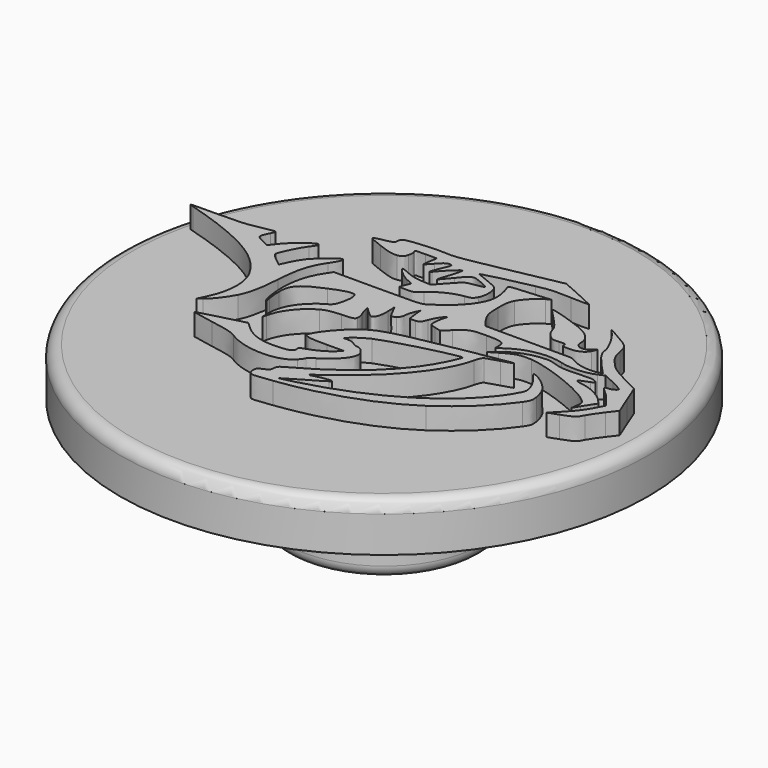
from build123d import *

# Parameters (mm, degrees)
F0_R     = 11
F1_DEPTH = 2
F2_DEPTH = 0.9
F3_R     = 0.5
F4_R     = 5.5
F4_R_2   = 4.1
F5_DEPTH = 1
F6_DEPTH = 4.5
F7_R     = 0.5


# Not quite as in the source:
# - ends of sketch curves that miss each other by under 0.0002 mm in the source are joined


with BuildPart() as f1:
    # F0 (on Top) → F1 (new body)
    with BuildSketch(Plane.XY):
        Circle(F0_R)
        with BuildLine():
            add(Edge.make_bspline(
                [(-0.1446416936, -5.6087199148), (-0.9458515916, -5.7124352464), (-0.9707127564, -5.7129654608), (-1.0555580465, -5.6281081884)],
                knots=[0, 0, 0, 0, 1, 1, 1, 1], degree=3))
            add(Edge.make_bspline(
                [(-1.0555580465, -5.6281081884), (-1.0923475378, -5.5913296808), (-1.122449937, -5.4928086532), (-1.122449937, -5.4091825567)],
                knots=[0, 0, 0, 0, 1, 1, 1, 1], degree=3))
            add(Edge.make_bspline(
                [(-1.122449937, -5.4091825567), (-1.122449937, -5.2853520285), (-1.0810722437, -5.2388798834), (-0.899480297, -5.1587625881)],
                knots=[0, 0, 0, 0, 1, 1, 1, 1], degree=3))
            add(Edge.make_bspline(
                [(-0.899480297, -5.1587625881), (-0.7144115017, -5.0771095682), (-0.676510657, -5.0333454108), (-0.676510657, -4.9012970585)],
                knots=[0, 0, 0, 0, 1, 1, 1, 1], degree=3))
            add(Edge.make_bspline(
                [(-0.676510657, -4.9012970585), (-0.676510657, -4.780510021), (-0.6345508262, -4.7193386547), (-0.5022458541, -4.6472474677)],
                knots=[0, 0, 0, 0, 1, 1, 1, 1], degree=3))
            add(Edge.make_bspline(
                [(-0.5022458541, -4.6472474677), (1.50229814, -3.5549698263), (2.7477118893, -2.4096058396), (3.4344503923, -1.0268046486)],
                knots=[0, 0, 0, 0, 1, 1, 1, 1], degree=3))
            add(Edge.make_bspline(
                [(3.4344503923, -1.0268046486), (3.5752288098, -0.7433336496), (3.6752156656, -0.4962107959), (3.6566421848, -0.477637315)],
                knots=[0, 0, 0, 0, 1, 1, 1, 1], degree=3))
            add(Edge.make_bspline(
                [(3.6566421848, -0.477637315), (3.5693335445, -0.3903286747), (1.0712418088, -1.0368078275), (0.5261294673, -1.287783972)],
                knots=[0, 0, 0, 0, 1, 1, 1, 1], degree=3))
            add(Edge.make_bspline(
                [(0.5261294673, -1.287783972), (0.3398824177, -1.3735339217), (0.0896451784, -1.5298223591), (-0.0299496255, -1.6350913886)],
                knots=[0, 0, 0, 0, 1, 1, 1, 1], degree=3))
            Line((-0.0299496255, -1.6350913886), (-0.2473984454, -1.8264898057))
            Line((-0.2473984454, -1.8264898057), (-0.0466608655, -1.8264898057))
            add(Edge.make_bspline(
                [(-0.0466608655, -1.8264898057), (0.0640461069, -1.8264898057), (0.2010431271, -1.8689918331), (0.2587905664, -1.921252402)],
                knots=[0, 0, 0, 0, 1, 1, 1, 1], degree=3))
            add(Edge.make_bspline(
                [(0.2587905664, -1.921252402), (0.3163822365, -1.9733691838), (0.4191060371, -2.0160120027), (0.4870663446, -2.0160120027)],
                knots=[0, 0, 0, 0, 1, 1, 1, 1], degree=3))
            add(Edge.make_bspline(
                [(0.4870663446, -2.0160120027), (0.6640281515, -2.0160120027), (0.8842758245, -2.2572365954), (0.8842758245, -2.4510564249)],
                knots=[0, 0, 0, 0, 1, 1, 1, 1], degree=3))
            add(Edge.make_bspline(
                [(0.8842758245, -2.4510564249), (0.8842758245, -2.7380232443), (0.4839549546, -3.1917260216), (-0.0403621979, -3.4989977566)],
                knots=[0, 0, 0, 0, 1, 1, 1, 1], degree=3))
            add(Edge.make_bspline(
                [(-0.0403621979, -3.4989977566), (-0.1756367701, -3.578275296), (-0.2863127885, -3.6649638551), (-0.2863127885, -3.6916423273)],
                knots=[0, 0, 0, 0, 1, 1, 1, 1], degree=3))
            add(Edge.make_bspline(
                [(-0.2863127885, -3.6916423273), (-0.2863127885, -3.7183287876), (-0.3627355577, -3.8271874986), (-0.456140166, -3.93356888)],
                knots=[0, 0, 0, 0, 1, 1, 1, 1], degree=3))
            add(Edge.make_bspline(
                [(-0.456140166, -3.93356888), (-0.9134805537, -4.4544481262), (-2.3035499758, -4.4471828907), (-3.1350909343, -3.9195636307)],
                knots=[0, 0, 0, 0, 1, 1, 1, 1], degree=3))
            add(Edge.make_bspline(
                [(-3.1350909343, -3.9195636307), (-3.3453703765, -3.7861403156), (-3.5546243382, -3.7284767521), (-4.2910652004, -3.6010116091)],
                knots=[0, 0, 0, 0, 1, 1, 1, 1], degree=3))
            add(Edge.make_bspline(
                [(-4.2910652004, -3.6010116091), (-4.7856344285, -3.5154104389), (-5.1805303362, -3.4356196599), (-5.1686099978, -3.4236993215)],
                knots=[0, 0, 0, 0, 1, 1, 1, 1], degree=3))
            add(Edge.make_bspline(
                [(-5.1686099978, -3.4236993215), (-5.1566896594, -3.4117789831), (-4.736138763, -3.2942860649), (-4.2340496767, -3.1626051682)],
                knots=[0, 0, 0, 0, 1, 1, 1, 1], degree=3))
            Line((-4.2340496767, -3.1626051682), (-3.3211632427, -2.9231859005))
            Line((-3.3211632427, -2.9231859005), (-3.0562896891, -3.1629905971))
            add(Edge.make_bspline(
                [(-3.0562896891, -3.1629905971), (-2.6786372328, -3.5049020086), (-2.2717710606, -3.6463704038), (-1.6665048453, -3.6462236213)],
                knots=[0, 0, 0, 0, 1, 1, 1, 1], degree=3))
            add(Edge.make_bspline(
                [(-1.6665048453, -3.6462236213), (-1.1267725325, -3.646088821), (-0.886751157, -3.5539014093), (-0.9359832129, -3.3656393453)],
                knots=[0, 0, 0, 0, 1, 1, 1, 1], degree=3))
            add(Edge.make_bspline(
                [(-0.9359832129, -3.3656393453), (-0.9574563975, -3.2834930562), (-0.9136353244, -3.2477490159), (-0.7222059532, -3.1912307554)],
                knots=[0, 0, 0, 0, 1, 1, 1, 1], degree=3))
            add(Edge.make_bspline(
                [(-0.7222059532, -3.1912307554), (-0.3904395105, -3.0932808816), (0.0106212631, -2.8695363896), (0.189959549, -2.6823477352)],
                knots=[0, 0, 0, 0, 1, 1, 1, 1], degree=3))
            Line((0.189959549, -2.6823477352), (0.339896397, -2.5258476115))
            Line((0.339896397, -2.5258476115), (-0.3494712106, -2.5337938381))
            add(Edge.make_bspline(
                [(-0.3494712106, -2.5337938381), (-0.7843888207, -2.5388104054), (-1.0967100741, -2.5167450981), (-1.1956315085, -2.4740204006)],
                knots=[0, 0, 0, 0, 1, 1, 1, 1], degree=3))
            Line((-1.1956315085, -2.4740204006), (-1.3524281928, -2.4063027336))
            Line((-1.3524281928, -2.4063027336), (-1.1956315085, -2.1137082523))
            add(Edge.make_bspline(
                [(-1.1956315085, -2.1137082523), (-1.1093942807, -1.9527806885), (-0.8507055634, -1.6305341408), (-0.6207672485, -1.3976052568)],
                knots=[0, 0, 0, 0, 1, 1, 1, 1], degree=3))
            add(Edge.make_bspline(
                [(-0.6207672485, -1.3976052568), (-0.0639103081, -0.8334970602), (0.2700089448, -0.6746044813), (1.4183654976, -0.4272988983)],
                knots=[0, 0, 0, 0, 1, 1, 1, 1], degree=3))
            add(Edge.make_bspline(
                [(1.4183654976, -0.4272988983), (2.5069855582, -0.1928592527), (5.1777165053, 0.2867241789), (5.2107435712, 0.2536991101)],
                knots=[0, 0, 0, 0, 1, 1, 1, 1], degree=3))
            add(Edge.make_bspline(
                [(5.2107435712, 0.2536991101), (5.2238481549, 0.2405955248), (5.0271006632, 0.1720550769), (4.7735073963, 0.1014097476)],
                knots=[0, 0, 0, 0, 1, 1, 1, 1], degree=3))
            add(Edge.make_bspline(
                [(4.7735073963, 0.1014097476), (4.519917125, 0.0307634198), (4.2732166454, -0.0465040978), (4.2252896558, -0.0702968456)],
                knots=[0, 0, 0, 0, 1, 1, 1, 1], degree=3))
            add(Edge.make_bspline(
                [(4.2252896558, -0.0702968456), (4.1773606692, -0.0940816052), (4.1074282836, -0.246870228), (4.0698829122, -0.4098128063)],
                knots=[0, 0, 0, 0, 1, 1, 1, 1], degree=3))
            add(Edge.make_bspline(
                [(4.0698829122, -0.4098128063), (3.7920096194, -1.6157819981), (2.5522544861, -3.104282581), (0.828534413, -4.3015157165)],
                knots=[0, 0, 0, 0, 1, 1, 1, 1], degree=3))
            add(Edge.make_bspline(
                [(0.828534413, -4.3015157165), (0.5985960981, -4.4612230882), (0.46063251, -4.5776415983), (0.5219506588, -4.5602264013)],
                knots=[0, 0, 0, 0, 1, 1, 1, 1], degree=3))
            add(Edge.make_bspline(
                [(0.5219506588, -4.5602264013), (0.7918407796, -4.4835729738), (1.146181775, -4.415694545), (1.274473693, -4.4160689902)],
                knots=[0, 0, 0, 0, 1, 1, 1, 1], degree=3))
            add(Edge.make_bspline(
                [(1.274473693, -4.4160689902), (1.4110583242, -4.416350573), (1.4116105061, -4.4183236496), (1.3023443988, -4.5022842505)],
                knots=[0, 0, 0, 0, 1, 1, 1, 1], degree=3))
            add(Edge.make_bspline(
                [(1.3023443988, -4.5022842505), (1.24102625, -4.549478326), (0.8968182412, -4.7542289599), (0.5374357155, -4.9572890986)],
                knots=[0, 0, 0, 0, 1, 1, 1, 1], degree=3))
            add(Edge.make_bspline(
                [(0.5374357155, -4.9572890986), (0.1780501943, -5.1603522328), (-0.1080289404, -5.3344512813), (-0.0983013531, -5.3441818641)],
                knots=[0, 0, 0, 0, 1, 1, 1, 1], degree=3))
            add(Edge.make_bspline(
                [(-0.0983013531, -5.3441818641), (-0.0885787585, -5.3539034602), (0.1678433172, -5.2977935946), (0.4715103929, -5.2194776305)],
                knots=[0, 0, 0, 0, 1, 1, 1, 1], degree=3))
            add(Edge.make_bspline(
                [(0.4715103929, -5.2194776305), (3.0454976789, -4.5556362023), (5.1017949934, -3.3605219274), (6.2564252508, -1.8573051486)],
                knots=[0, 0, 0, 0, 1, 1, 1, 1], degree=3))
            add(Edge.make_bspline(
                [(6.2564252508, -1.8573051486), (6.5109711063, -1.5259081585), (6.7374375653, -1.1222821855), (6.736913342, -1.000934978)],
                knots=[0, 0, 0, 0, 1, 1, 1, 1], degree=3))
            add(Edge.make_bspline(
                [(6.736913342, -1.000934978), (6.7360685936, -0.7892486203), (6.5920549695, -0.4739517757), (6.3742446852, -0.2065379857)],
                knots=[0, 0, 0, 0, 1, 1, 1, 1], degree=3))
            add(Edge.make_bspline(
                [(6.3742446852, -0.2065379857), (6.1437541884, 0.0764417411), (6.1380196848, 0.0914554962), (6.279752688, 0.0408944093)],
                knots=[0, 0, 0, 0, 1, 1, 1, 1], degree=3))
            add(Edge.make_bspline(
                [(6.279752688, 0.0408944093), (6.5494820471, -0.0553250284), (6.949754988, -0.389688623), (7.0979643955, -0.6425889167)],
                knots=[0, 0, 0, 0, 1, 1, 1, 1], degree=3))
            add(Edge.make_bspline(
                [(7.0979643955, -0.6425889167), (7.1776253669, -0.7785225125), (7.2576268338, -1.0148952939), (7.2757439908, -1.1678586578)],
                knots=[0, 0, 0, 0, 1, 1, 1, 1], degree=3))
            add(Edge.make_bspline(
                [(7.2757439908, -1.1678586578), (7.3053671001, -1.4179800687), (7.2904541956, -1.4724753265), (7.1275565507, -1.7092305413)],
                knots=[0, 0, 0, 0, 1, 1, 1, 1], degree=3))
            add(Edge.make_bspline(
                [(7.1275565507, -1.7092305413), (6.6189900615, -2.4484103454), (5.7579408236, -3.2670244567), (4.8419829404, -3.8821650418)],
                knots=[0, 0, 0, 0, 1, 1, 1, 1], degree=3))
            add(Edge.make_bspline(
                [(4.8419829404, -3.8821650418), (3.5579224516, -4.7445183475), (1.7823811587, -5.3592755008), (-0.1446416936, -5.6087199148)],
                knots=[0, 0, 0, 0, 1, 1, 1, 1], degree=3))
        make_face(mode=Mode.SUBTRACT)
        with BuildLine():
            Line((-5.7022802923, -2.6431488137), (-5.5649287973, -2.3713874653))
            add(Edge.make_bspline(
                [(-5.5649287973, -2.3713874653), (-5.1782986427, -1.606399899), (-5.1432675461, -0.7986327165), (-5.4701272588, -0.1853803337)],
                knots=[0, 0, 0, 0, 1, 1, 1, 1], degree=3))
            add(Edge.make_bspline(
                [(-5.4701272588, -0.1853803337), (-6.0299777637, 0.8650043778), (-7.2980339651, 1.6002160612), (-9.8461316102, 2.351794495)],
                knots=[0, 0, 0, 0, 1, 1, 1, 1], degree=3))
            add(Edge.make_bspline(
                [(-9.8461316102, 2.351794495), (-10.1136402595, 2.4306965908), (-10.0789107161, 2.4340446302), (-8.9821237559, 2.4350960723)],
                knots=[0, 0, 0, 0, 1, 1, 1, 1], degree=3))
            add(Edge.make_bspline(
                [(-8.9821237559, 2.4350960723), (-8.045196941, 2.4359418192), (-7.7404245031, 2.4569077553), (-7.2897791957, 2.5512669493)],
                knots=[0, 0, 0, 0, 1, 1, 1, 1], degree=3))
            add(Edge.make_bspline(
                [(-7.2897791957, 2.5512669493), (-6.5593843755, 2.7041943664), (-6.5796124049, 2.7074125982), (-6.6988377562, 2.4573101591)],
                knots=[0, 0, 0, 0, 1, 1, 1, 1], degree=3))
            add(Edge.make_bspline(
                [(-6.6988377562, 2.4573101591), (-6.89532064, 2.0451488325), (-6.8929451596, 2.034899019), (-6.5635292343, 1.8733383931)],
                knots=[0, 0, 0, 0, 1, 1, 1, 1], degree=3))
            Line((-6.5635292343, 1.8733383931), (-6.2630214776, 1.7259567591))
            Line((-6.2630214776, 1.7259567591), (-6.0136040237, 2.0471358884))
            add(Edge.make_bspline(
                [(-6.0136040237, 2.0471358884), (-5.7948701078, 2.3288015622), (-5.1558868489, 2.8335736733), (-5.0180650507, 2.8335736733)],
                knots=[0, 0, 0, 0, 1, 1, 1, 1], degree=3))
            add(Edge.make_bspline(
                [(-5.0180650507, 2.8335736733), (-4.9251397323, 2.8335736733), (-4.9686612492, 2.7102753566), (-5.1362958756, 2.498619953)],
                knots=[0, 0, 0, 0, 1, 1, 1, 1], degree=3))
            add(Edge.make_bspline(
                [(-5.1362958756, 2.498619953), (-5.2962448893, 2.2966681722), (-5.5952598577, 1.7044915628), (-5.6567607358, 1.4678861261)],
                knots=[0, 0, 0, 0, 1, 1, 1, 1], degree=3))
            add(Edge.make_bspline(
                [(-5.6567607358, 1.4678861261), (-5.6787701258, 1.3832175741), (-5.6161079684, 1.3013758338), (-5.3962746815, 1.1276602173)],
                knots=[0, 0, 0, 0, 1, 1, 1, 1], degree=3))
            Line((-5.3962746815, 1.1276602173), (-5.1068135577, 0.8989191284))
            Line((-5.1068135577, 0.8989191284), (-4.9754252274, 1.1966290305))
            add(Edge.make_bspline(
                [(-4.9754252274, 1.1966290305), (-4.9031612963, 1.3603714238), (-4.7551016669, 1.6084927981), (-4.6464007222, 1.7480140782)],
                knots=[0, 0, 0, 0, 1, 1, 1, 1], degree=3))
            add(Edge.make_bspline(
                [(-4.6464007222, 1.7480140782), (-4.457158111, 1.990915187), (-3.8417269564, 2.4991192133), (-3.7368173943, 2.4991192133)],
                knots=[0, 0, 0, 0, 1, 1, 1, 1], degree=3))
            add(Edge.make_bspline(
                [(-3.7368173943, 2.4991192133), (-3.630204356, 2.4991192133), (-3.6960088577, 2.3192117708), (-3.9252232452, 1.98404237)],
                knots=[0, 0, 0, 0, 1, 1, 1, 1], degree=3))
            add(Edge.make_bspline(
                [(-3.9252232452, 1.98404237), (-4.2768532573, 1.4698641953), (-4.4097972826, 1.0036040235), (-4.4696076653, 0.0747901881)],
                knots=[0, 0, 0, 0, 1, 1, 1, 1], degree=3))
            add(Edge.make_bspline(
                [(-4.4696076653, 0.0747901881), (-4.5228038479, -0.7513058377), (-4.6142214003, -1.2006301024), (-4.8074550982, -1.5857105531)],
                knots=[0, 0, 0, 0, 1, 1, 1, 1], degree=3))
            add(Edge.make_bspline(
                [(-4.8074550982, -1.5857105531), (-4.9767123204, -1.9230078011), (-5.3257272072, -2.3750200831), (-5.5282830929, -2.5192503862)],
                knots=[0, 0, 0, 0, 1, 1, 1, 1], degree=3))
            Line((-5.5282830929, -2.5192503862), (-5.7022802923, -2.6431488137))
        make_face(mode=Mode.SUBTRACT)
        with BuildLine():
            add(Edge.make_bspline(
                [(-3.1826055349, -2.1466654218), (-3.2273083016, -2.3726186412), (-3.2285933976, -2.3697898324), (-3.2345485742, -2.0320442487)],
                knots=[0, 0, 0, 0, 1, 1, 1, 1], degree=3))
            add(Edge.make_bspline(
                [(-3.2345485742, -2.0320442487), (-3.2428922119, -1.5598289003), (-3.0794623556, -1.144967574), (-2.7379263878, -0.7712722547)],
                knots=[0, 0, 0, 0, 1, 1, 1, 1], degree=3))
            add(Edge.make_bspline(
                [(-2.7379263878, -0.7712722547), (-2.5883869509, -0.6076506825), (-2.3511244877, -0.4131658383), (-2.2106785775, -0.3390826028)],
                knots=[0, 0, 0, 0, 1, 1, 1, 1], degree=3))
            add(Edge.make_bspline(
                [(-2.2106785775, -0.3390826028), (-1.9900255052, -0.2226910528), (-1.9441784339, -0.1670265274), (-1.8733383931, 0.0705065349)],
                knots=[0, 0, 0, 0, 1, 1, 1, 1], degree=3))
            add(Edge.make_bspline(
                [(-1.8733383931, 0.0705065349), (-1.7810701012, 0.379900126), (-1.7690279433, 0.6495306316), (-1.8423113639, 0.7652651551)],
                knots=[0, 0, 0, 0, 1, 1, 1, 1], degree=3))
            add(Edge.make_bspline(
                [(-1.8423113639, 0.7652651551), (-1.915135465, 0.8802727556), (-2.2383745422, 0.816925613), (-2.8087354745, 0.5758667747)],
                knots=[0, 0, 0, 0, 1, 1, 1, 1], degree=3))
            add(Edge.make_bspline(
                [(-2.8087354745, 0.5758667747), (-3.6978860763, 0.2000745622), (-3.9104421455, -0.0250988127), (-3.9082384106, -0.5888914768)],
                knots=[0, 0, 0, 0, 1, 1, 1, 1], degree=3))
            add(Edge.make_bspline(
                [(-3.9082384106, -0.5888914768), (-3.9073936622, -0.7759702939), (-3.8851026893, -1.0229263947), (-3.8584551713, -1.1376773755)],
                knots=[0, 0, 0, 0, 1, 1, 1, 1], degree=3))
            add(Edge.make_bspline(
                [(-3.8584551713, -1.1376773755), (-3.8317966695, -1.2524313518), (-3.8295050648, -1.3342641053), (-3.8533547283, -1.3195319331)],
                knots=[0, 0, 0, 0, 1, 1, 1, 1], degree=3))
            add(Edge.make_bspline(
                [(-3.8533547283, -1.3195319331), (-3.9460284195, -1.262254797), (-4.0349576587, -0.5400258778), (-4.0068143568, -0.0731855656)],
                knots=[0, 0, 0, 0, 1, 1, 1, 1], degree=3))
            add(Edge.make_bspline(
                [(-4.0068143568, -0.0731855656), (-3.9745192065, 0.4625536635), (-3.8277975946, 0.9190772614), (-3.5521589909, 1.34146244)],
                knots=[0, 0, 0, 0, 1, 1, 1, 1], degree=3))
            Line((-3.5521589909, 1.34146244), (-3.3800270279, 1.605237621))
            Line((-3.3800270279, 1.605237621), (-1.5749804512, 1.6063649508))
            add(Edge.make_bspline(
                [(-1.5749804512, 1.6063649508), (0.1824237143, 1.6072096991), (0.2353922342, 1.6105916883), (0.4317453103, 1.7293637113)],
                knots=[0, 0, 0, 0, 1, 1, 1, 1], degree=3))
            add(Edge.make_bspline(
                [(0.4317453103, 1.7293637113), (1.1839348387, 2.1843775461), (1.7192626773, 2.7824903602), (1.8342672823, 3.296380961)],
                knots=[0, 0, 0, 0, 1, 1, 1, 1], degree=3))
            add(Edge.make_bspline(
                [(1.8342672823, 3.296380961), (1.8976333967, 3.5795414201), (1.8476534489, 3.9427512751), (1.6977275845, 4.2887735957)],
                knots=[0, 0, 0, 0, 1, 1, 1, 1], degree=3))
            add(Edge.make_bspline(
                [(1.6977275845, 4.2887735957), (1.6641503338, 4.3662587908), (1.7354407074, 4.3831867098), (2.2331842323, 4.4159232062)],
                knots=[0, 0, 0, 0, 1, 1, 1, 1], degree=3))
            add(Edge.make_bspline(
                [(2.2331842323, 4.4159232062), (2.5489883254, 4.4366924337), (2.9327956623, 4.4666959794), (3.086088538, 4.4825954222)],
                knots=[0, 0, 0, 0, 1, 1, 1, 1], degree=3))
            Line((3.086088538, 4.4825954222), (3.3647995895, 4.5115035908))
            Line((3.3647995895, 4.5115035908), (3.197573358, 4.4187190637))
            add(Edge.make_bspline(
                [(3.197573358, 4.4187190637), (2.94582336, 4.2790400173), (2.617633618, 3.9481053423), (2.4825337869, 3.6977023485)],
                knots=[0, 0, 0, 0, 1, 1, 1, 1], degree=3))
            add(Edge.make_bspline(
                [(2.4825337869, 3.6977023485), (2.3847836171, 3.5165237893), (2.3622000777, 3.3807060219), (2.3620483026, 2.9730530156)],
                knots=[0, 0, 0, 0, 1, 1, 1, 1], degree=3))
            add(Edge.make_bspline(
                [(2.3620483026, 2.9730530156), (2.3618256325, 2.4453568695), (2.41018598, 2.2942637347), (2.7053087154, 1.9000108742)],
                knots=[0, 0, 0, 0, 1, 1, 1, 1], degree=3))
            Line((2.7053087154, 1.9000108742), (2.8409217861, 1.7188502884))
            Line((2.8409217861, 1.7188502884), (4.6302206951, 1.7188502884))
            Line((4.6302206951, 1.7188502884), (6.4195196042, 1.7188502884))
            Line((6.4195196042, 1.7188502884), (6.7180492917, 1.5727906956))
            add(Edge.make_bspline(
                [(6.7180492917, 1.5727906956), (7.0281927717, 1.4210525165), (7.4539319809, 1.3736078123), (7.7581682133, 1.456881431)],
                knots=[0, 0, 0, 0, 1, 1, 1, 1], degree=3))
            Line((7.7581682133, 1.456881431), (7.9151166727, 1.4998397824))
            Line((7.9151166727, 1.4998397824), (7.5287281601, 1.9135827656))
            add(Edge.make_bspline(
                [(7.5287281601, 1.9135827656), (7.1549649414, 2.3138047819), (6.9601815397, 2.6170514805), (6.9601815397, 2.7987253059)],
                knots=[0, 0, 0, 0, 1, 1, 1, 1], degree=3))
            add(Edge.make_bspline(
                [(6.9601815397, 2.7987253059), (6.9601815397, 2.972371026), (6.6704358375, 3.5362984904), (6.4415010357, 3.8082285888)],
                knots=[0, 0, 0, 0, 1, 1, 1, 1], degree=3))
            Line((6.4415010357, 3.8082285888), (6.207661501, 4.0859810606))
            Line((6.207661501, 4.0859810606), (6.542115961, 3.8987045363))
            add(Edge.make_bspline(
                [(6.542115961, 3.8987045363), (7.2772088204, 3.4870953915), (7.3103327428, 3.4543269425), (7.3902153858, 3.0596347329)],
                knots=[0, 0, 0, 0, 1, 1, 1, 1], degree=3))
            add(Edge.make_bspline(
                [(7.3902153858, 3.0596347329), (7.4702318305, 2.6643044688), (7.5095655522, 2.591133881), (7.8468518165, 2.2102412255)],
                knots=[0, 0, 0, 0, 1, 1, 1, 1], degree=3))
            add(Edge.make_bspline(
                [(7.8468518165, 2.2102412255), (8.0192823371, 2.0155167365), (8.2442590034, 1.8643287421), (8.7315300447, 1.6157210884)],
                knots=[0, 0, 0, 0, 1, 1, 1, 1], degree=3))
            Line((8.7315300447, 1.6157210884), (9.3849758754, 1.2823320498))
            Line((9.3849758754, 1.2823320498), (9.6850812283, 0.5328075728))
            Line((9.6850812283, 0.5328075728), (9.9851865812, -0.2167139087))
            Line((9.9851865812, -0.2167139087), (9.6973230903, -0.5922924378))
            add(Edge.make_bspline(
                [(9.6973230903, -0.5922924378), (9.5389966726, -0.7988603792), (9.3618850876, -1.061119806), (9.3037402371, -1.1750899436)],
                knots=[0, 0, 0, 0, 1, 1, 1, 1], degree=3))
            add(Edge.make_bspline(
                [(9.3037402371, -1.1750899436), (9.1676618559, -1.4418267366), (9.1317550567, -1.4671102756), (8.6324528412, -1.647763613)],
                knots=[0, 0, 0, 0, 1, 1, 1, 1], degree=3))
            Line((8.6324528412, -1.647763613), (8.2143842669, -1.7990254978))
            Line((8.2143842669, -1.7990254978), (8.6112442646, -1.3918397991))
            add(Edge.make_bspline(
                [(8.6112442646, -1.3918397991), (8.8528183396, -1.1439790387), (9.0868915281, -0.8334381475), (9.2094619233, -0.5981847076)],
                knots=[0, 0, 0, 0, 1, 1, 1, 1], degree=3))
            Line((9.2094619233, -0.5981847076), (9.4108255756, -0.2117153148))
            Line((9.4108255756, -0.2117153148), (9.1888374813, 0.0823060523))
            add(Edge.make_bspline(
                [(9.1888374813, 0.0823060523), (9.0667453774, 0.2440164563), (8.8790684464, 0.4463666468), (8.7717834039, 0.531969814)],
                knots=[0, 0, 0, 0, 1, 1, 1, 1], degree=3))
            add(Edge.make_bspline(
                [(8.7717834039, 0.531969814), (8.5484503024, 0.7101697864), (8.5280525245, 0.7712283198), (8.6918608201, 0.7712283198)],
                knots=[0, 0, 0, 0, 1, 1, 1, 1], degree=3))
            add(Edge.make_bspline(
                [(8.6918608201, 0.7712283198), (8.8366912341, 0.7712283198), (9.0226507097, 0.8683663965), (9.0226507097, 0.9440193064)],
                knots=[0, 0, 0, 0, 1, 1, 1, 1], degree=3))
            add(Edge.make_bspline(
                [(9.0226507097, 0.9440193064), (9.0226507097, 0.975578547), (8.8107626508, 1.0992942453), (8.5517893551, 1.2189399738)],
                knots=[0, 0, 0, 0, 1, 1, 1, 1], degree=3))
            Line((8.5517893551, 1.2189399738), (8.0809299976, 1.4364786605))
            Line((8.0809299976, 1.4364786605), (7.8225298528, 1.3221760155))
            add(Edge.make_bspline(
                [(7.8225298528, 1.3221760155), (7.4465878622, 1.1558804052), (6.8497881026, 1.1243601068), (6.4027584382, 1.2471931129)],
                knots=[0, 0, 0, 0, 1, 1, 1, 1], degree=3))
            add(Edge.make_bspline(
                [(6.4027584382, 1.2471931129), (5.7239831366, 1.4337057689), (4.9652213459, 1.3074937693), (4.3542266181, 0.9064409838)],
                knots=[0, 0, 0, 0, 1, 1, 1, 1], degree=3))
            Line((4.3542266181, 0.9064409838), (4.0615782167, 0.7143485949))
            Line((4.0615782167, 0.7143485949), (4.0615782167, 0.9113946443))
            add(Edge.make_bspline(
                [(4.0615782167, 0.9113946443), (4.0615782167, 1.1653913135), (3.9422340414, 1.2135369791), (3.2937588461, 1.2211656761)],
                knots=[0, 0, 0, 0, 1, 1, 1, 1], degree=3))
            add(Edge.make_bspline(
                [(3.2937588461, 1.2211656761), (2.7002222516, 1.2281543215), (2.5762169824, 1.1833277382), (2.1971526181, 0.8248219136)],
                knots=[0, 0, 0, 0, 1, 1, 1, 1], degree=3))
            Line((2.1971526181, 0.8248219136), (1.8997892026, 0.5435915947))
            Line((1.8997892026, 0.5435915947), (1.6428678667, 0.6082857415))
            add(Edge.make_bspline(
                [(1.6428678667, 0.6082857415), (1.3964050351, 0.6703447926), (1.3859465308, 0.6812336592), (1.3859465308, 0.8757634368)],
                knots=[0, 0, 0, 0, 1, 1, 1, 1], degree=3))
            add(Edge.make_bspline(
                [(1.3859465308, 0.8757634368), (1.3859465308, 0.9872961857), (1.4102385388, 1.1661771492), (1.439901589, 1.2732774654)],
                knots=[0, 0, 0, 0, 1, 1, 1, 1], degree=3))
            Line((1.439901589, 1.2732774654), (1.4938586442, 1.4680099426))
            Line((1.4938586442, 1.4680099426), (1.3583134729, 1.3139611869))
            add(Edge.make_bspline(
                [(1.3583134729, 1.3139611869), (1.2837619312, 1.2292367178), (1.1791049948, 1.0369815701), (1.1257400622, 0.886728191)],
                knots=[0, 0, 0, 0, 1, 1, 1, 1], degree=3))
            add(Edge.make_bspline(
                [(1.1257400622, 0.886728191), (1.0377833821, 0.6390781184), (1.0102332014, 0.6112273831), (0.8310676597, 0.5888105966)],
                knots=[0, 0, 0, 0, 1, 1, 1, 1], degree=3))
            add(Edge.make_bspline(
                [(0.8310676597, 0.5888105966), (0.7223647179, 0.5751987644), (0.6210218712, 0.5750020559), (0.6058633307, 0.5882464325)],
                knots=[0, 0, 0, 0, 1, 1, 1, 1], degree=3))
            add(Edge.make_bspline(
                [(0.6058633307, 0.5882464325), (0.5907027931, 0.6016046405), (0.5647033149, 0.7548246241), (0.5480739535, 0.9287259655)],
                knots=[0, 0, 0, 0, 1, 1, 1, 1], degree=3))
            Line((0.5480739535, 0.9287259655), (0.5178447422, 1.2449104949))
            Line((0.5178447422, 1.2449104949), (0.4223412437, 1.0290712902))
            add(Edge.make_bspline(
                [(0.4223412437, 1.0290712902), (0.3698160669, 0.9103581799), (0.3268407408, 0.7439237752), (0.3268407408, 0.6592192765)],
                knots=[0, 0, 0, 0, 1, 1, 1, 1], degree=3))
            add(Edge.make_bspline(
                [(0.3268407408, 0.6592192765), (0.3268407408, 0.5550785752), (0.2801539137, 0.4746197859), (0.18264938, 0.4107324437)],
                knots=[0, 0, 0, 0, 1, 1, 1, 1], degree=3))
            add(Edge.make_bspline(
                [(0.18264938, 0.4107324437), (0.0139333558, 0.3001862331), (0.0187402338, 0.2968801315), (-0.154935442, 0.6429084433)],
                knots=[0, 0, 0, 0, 1, 1, 1, 1], degree=3))
            Line((-0.154935442, 0.6429084433), (-0.2892214788, 0.9104560349))
            Line((-0.2892214788, 0.9104560349), (-0.2764553935, 0.5481318677))
            add(Edge.make_bspline(
                [(-0.2764553935, 0.5481318677), (-0.2637182653, 0.1864916871), (-0.3497927343, -0.0650356408), (-0.4862675282, -0.0650356408)],
                knots=[0, 0, 0, 0, 1, 1, 1, 1], degree=3))
            add(Edge.make_bspline(
                [(-0.4862675282, -0.0650356408), (-0.5201772862, -0.0650356408), (-0.6405948711, 0.0249700035), (-0.7538660444, 0.1349750161)],
                knots=[0, 0, 0, 0, 1, 1, 1, 1], degree=3))
            Line((-0.7538660444, 0.1349750161), (-0.9598089119, 0.3349856729))
            Line((-0.9598089119, 0.3349856729), (-0.9231691986, 0.1767840702))
            add(Edge.make_bspline(
                [(-0.9231691986, 0.1767840702), (-0.9030200524, 0.089770992), (-0.852143433, -0.0536025805), (-0.8101147043, -0.1418278626)],
                knots=[0, 0, 0, 0, 1, 1, 1, 1], degree=3))
            add(Edge.make_bspline(
                [(-0.8101147043, -0.1418278626), (-0.7680859756, -0.2300491507), (-0.7479038782, -0.3588373334), (-0.7652681506, -0.4280198301)],
                knots=[0, 0, 0, 0, 1, 1, 1, 1], degree=3))
            add(Edge.make_bspline(
                [(-0.7652681506, -0.4280198301), (-0.7945727319, -0.5447768386), (-0.8335300114, -0.5555368962), (-1.3080329704, -0.5779227285)],
                knots=[0, 0, 0, 0, 1, 1, 1, 1], degree=3))
            add(Edge.make_bspline(
                [(-1.3080329704, -0.5779227285), (-1.7192726625, -0.5973110021), (-1.873721825, -0.6303869955), (-2.0979396157, -0.7470112008)],
                knots=[0, 0, 0, 0, 1, 1, 1, 1], degree=3))
            add(Edge.make_bspline(
                [(-2.0979396157, -0.7470112008), (-2.6179451564, -1.0174874533), (-3.0761961949, -1.6088123246), (-3.1826055349, -2.1466654218)],
                knots=[0, 0, 0, 0, 1, 1, 1, 1], degree=3))
        make_face(mode=Mode.SUBTRACT)
        with BuildLine():
            add(Edge.make_bspline(
                [(-0.7601786914, 2.1089632826), (-0.9287659064, 2.1089632826), (-1.0666975418, 2.1223204921), (-1.0666975418, 2.1386233372)],
                knots=[0, 0, 0, 0, 1, 1, 1, 1], degree=3))
            add(Edge.make_bspline(
                [(-1.0666975418, 2.1386233372), (-1.0667065285, 2.1549002208), (-1.0304123033, 2.2551097467), (-0.9860540262, 2.3612774447)],
                knots=[0, 0, 0, 0, 1, 1, 1, 1], degree=3))
            Line((-0.9860540262, 2.3612774447), (-0.9053985283, 2.5543074444))
            Line((-0.9053985283, 2.5543074444), (-1.1815583598, 2.6731084245))
            add(Edge.make_bspline(
                [(-1.1815583598, 2.6731084245), (-1.4198692696, 2.7756255314), (-1.8358329625, 3.1421325012), (-1.7787086001, 3.1992568637)],
                knots=[0, 0, 0, 0, 1, 1, 1, 1], degree=3))
            add(Edge.make_bspline(
                [(-1.7787086001, 3.1992568637), (-1.7679715085, 3.2099939552), (-1.6221915016, 3.1531092377), (-1.4547545822, 3.0728451599)],
                knots=[0, 0, 0, 0, 1, 1, 1, 1], degree=3))
            add(Edge.make_bspline(
                [(-1.4547545822, 3.0728451599), (-1.2468955538, 2.9732047907), (-1.0255914461, 2.9188473287), (-0.7571322051, 2.9014850533)],
                knots=[0, 0, 0, 0, 1, 1, 1, 1], degree=3))
            Line((-0.7571322051, 2.9014850533), (-0.3639417705, 2.876066714))
            Line((-0.3639417705, 2.876066714), (0.0117775499, 3.295870717))
            add(Edge.make_bspline(
                [(0.0117775499, 3.295870717), (0.3656811933, 3.6912938436), (0.4043508989, 3.7179832995), (0.6776959009, 3.7554917257)],
                knots=[0, 0, 0, 0, 1, 1, 1, 1], degree=3))
            add(Edge.make_bspline(
                [(0.6776959009, 3.7554917257), (1.1847356522, 3.8250666409), (1.2134970383, 3.857228988), (0.8922530052, 3.9954232344)],
                knots=[0, 0, 0, 0, 1, 1, 1, 1], degree=3))
            add(Edge.make_bspline(
                [(0.8922530052, 3.9954232344), (0.3413192888, 4.2324290778), (0.3429338966, 4.2328834047), (-0.0590175574, 3.7289680242)],
                knots=[0, 0, 0, 0, 1, 1, 1, 1], degree=3))
            add(Edge.make_bspline(
                [(-0.0590175574, 3.7289680242), (-0.2559178228, 3.4821217606), (-0.4251021531, 3.2882430185), (-0.434984511, 3.2981253764)],
                knots=[0, 0, 0, 0, 1, 1, 1, 1], degree=3))
            add(Edge.make_bspline(
                [(-0.434984511, 3.2981253764), (-0.4448758556, 3.3080167211), (-0.3795626261, 3.5332100663), (-0.2898635276, 3.7985738936)],
                knots=[0, 0, 0, 0, 1, 1, 1, 1], degree=3))
            add(Edge.make_bspline(
                [(-0.2898635276, 3.7985738936), (-0.1978578466, 4.0707606117), (-0.1493676913, 4.2950183432), (-0.1786073688, 4.3130875712)],
                knots=[0, 0, 0, 0, 1, 1, 1, 1], degree=3))
            add(Edge.make_bspline(
                [(-0.1786073688, 4.3130875712), (-0.2249976352, 4.3417580919), (-0.8443200245, 3.7271587049), (-0.8901890632, 3.606932836)],
                knots=[0, 0, 0, 0, 1, 1, 1, 1], degree=3))
            add(Edge.make_bspline(
                [(-0.8901890632, 3.606932836), (-0.9004189063, 3.5801335428), (-0.930716017, 3.5582309944), (-0.9575352806, 3.5582309944)],
                knots=[0, 0, 0, 0, 1, 1, 1, 1], degree=3))
            add(Edge.make_bspline(
                [(-0.9575352806, 3.5582309944), (-0.9843625324, 3.5582309944), (-0.9320879842, 3.7236169525), (-0.8414063415, 3.9257524611)],
                knots=[0, 0, 0, 0, 1, 1, 1, 1], degree=3))
            add(Edge.make_bspline(
                [(-0.8414063415, 3.9257524611), (-0.6417561505, 4.3707331614), (-0.6403023046, 4.3943681429), (-0.8125490974, 4.3943681429)],
                knots=[0, 0, 0, 0, 1, 1, 1, 1], degree=3))
            add(Edge.make_bspline(
                [(-0.8125490974, 4.3943681429), (-0.9073176848, 4.3943681429), (-1.0199607887, 4.3097225569), (-1.1838579526, 4.1153475501)],
                knots=[0, 0, 0, 0, 1, 1, 1, 1], degree=3))
            add(Edge.make_bspline(
                [(-1.1838579526, 4.1153475501), (-1.3132572299, 3.9618879215), (-1.4292343939, 3.8464359793), (-1.4415830976, 3.858784683)],
                knots=[0, 0, 0, 0, 1, 1, 1, 1], degree=3))
            add(Edge.make_bspline(
                [(-1.4415830976, 3.858784683), (-1.4539258102, 3.8711273956), (-1.4407373507, 4.0092317751), (-1.412337429, 4.1656729861)],
                knots=[0, 0, 0, 0, 1, 1, 1, 1], degree=3))
            Line((-1.412337429, 4.1656729861), (-1.3606400258, 4.4501095544))
            Line((-1.3606400258, 4.4501095544), (-1.8336631774, 4.4501095544))
            add(Edge.make_bspline(
                [(-1.8336631774, 4.4501095544), (-2.2365392614, 4.4501095544), (-2.2969217964, 4.4383300074), (-2.2408289057, 4.3707501362)],
                knots=[0, 0, 0, 0, 1, 1, 1, 1], degree=3))
            add(Edge.make_bspline(
                [(-2.2408289057, 4.3707501362), (-2.1920262135, 4.3119462622), (-2.1903177449, 4.2343761929), (-2.2342346759, 4.0712538809)],
                knots=[0, 0, 0, 0, 1, 1, 1, 1], degree=3))
            add(Edge.make_bspline(
                [(-2.2342346759, 4.0712538809), (-2.287867212, 3.8720739931), (-2.3144697966, 3.8477630132), (-2.5136237229, 3.8159191941)],
                knots=[0, 0, 0, 0, 1, 1, 1, 1], degree=3))
            add(Edge.make_bspline(
                [(-2.5136237229, 3.8159191941), (-2.690789228, 3.7875891689), (-2.8557518133, 3.82626187), (-3.3590890504, 4.0141744519)],
                knots=[0, 0, 0, 0, 1, 1, 1, 1], degree=3))
            add(Edge.make_bspline(
                [(-3.3590890504, 4.0141744519), (-4.0391544406, 4.2680552927), (-4.0421330274, 4.2806007049), (-3.4496858189, 4.3957291265)],
                knots=[0, 0, 0, 0, 1, 1, 1, 1], degree=3))
            add(Edge.make_bspline(
                [(-3.4496858189, 4.3957291265), (-3.1701250265, 4.4500556343), (-3.1291677103, 4.4744464959), (-3.1291677103, 4.586593335)],
                knots=[0, 0, 0, 0, 1, 1, 1, 1], degree=3))
            add(Edge.make_bspline(
                [(-3.1291677103, 4.586593335), (-3.1291677103, 4.6573095593), (-3.0938969687, 4.7444434585), (-3.0507888393, 4.780218453)],
                knots=[0, 0, 0, 0, 1, 1, 1, 1], degree=3))
            add(Edge.make_bspline(
                [(-3.0507888393, 4.780218453), (-2.9464474354, 4.8668141496), (-1.7395655958, 4.9643436463), (-1.3155368523, 4.9204466857)],
                knots=[0, 0, 0, 0, 1, 1, 1, 1], degree=3))
            add(Edge.make_bspline(
                [(-1.3155368523, 4.9204466857), (-1.0322445885, 4.891120137), (-0.6614969019, 4.9491152093), (1.030712858, 5.2874698906)],
                knots=[0, 0, 0, 0, 1, 1, 1, 1], degree=3))
            Line((1.030712858, 5.2874698906), (3.040501082, 5.689320494))
            Line((3.040501082, 5.689320494), (3.7600839217, 5.3718618524))
            add(Edge.make_bspline(
                [(3.7600839217, 5.3718618524), (4.1558535349, 5.1972605481), (4.4972736743, 5.0375881246), (4.5187917923, 5.0170325805)],
                knots=[0, 0, 0, 0, 1, 1, 1, 1], degree=3))
            add(Edge.make_bspline(
                [(4.5187917923, 5.0170325805), (4.5403218925, 4.9964890186), (4.2016776403, 4.9962074358), (3.7662697566, 5.0164694149)],
                knots=[0, 0, 0, 0, 1, 1, 1, 1], degree=3))
            add(Edge.make_bspline(
                [(3.7662697566, 5.0164694149), (3.0626452724, 5.0491559852), (2.9064467019, 5.0388163049), (2.3614561799, 4.9235670624)],
                knots=[0, 0, 0, 0, 1, 1, 1, 1], degree=3))
            add(Edge.make_bspline(
                [(2.3614561799, 4.9235670624), (1.0690969867, 4.6502470234), (0.3840020485, 4.4824636175), (0.4243223085, 4.4491509747)],
                knots=[0, 0, 0, 0, 1, 1, 1, 1], degree=3))
            add(Edge.make_bspline(
                [(0.4243223085, 4.4491509747), (0.447374154, 4.4301011995), (0.641805078, 4.3465719595), (0.8564131069, 4.2634950493)],
                knots=[0, 0, 0, 0, 1, 1, 1, 1], degree=3))
            add(Edge.make_bspline(
                [(0.8564131069, 4.2634950493), (1.0710221343, 4.1804191376), (1.2946757609, 4.0760078372), (1.3534237178, 4.0314718234)],
                knots=[0, 0, 0, 0, 1, 1, 1, 1], degree=3))
            add(Edge.make_bspline(
                [(1.3534237178, 4.0314718234), (1.5080645962, 3.9142325295), (1.5360950652, 3.4260598241), (1.4029872826, 3.1682418167)],
                knots=[0, 0, 0, 0, 1, 1, 1, 1], degree=3))
            add(Edge.make_bspline(
                [(1.4029872826, 3.1682418167), (1.3123905141, 2.9927618143), (1.2717706979, 2.9689920325), (0.9957686327, 2.9299169276)],
                knots=[0, 0, 0, 0, 1, 1, 1, 1], degree=3))
            add(Edge.make_bspline(
                [(0.9957686327, 2.9299169276), (0.5841305308, 2.871645265), (0.0724436648, 2.6228708583), (-0.2166899442, 2.3404373222)],
                knots=[0, 0, 0, 0, 1, 1, 1, 1], degree=3))
            add(Edge.make_bspline(
                [(-0.2166899442, 2.3404373222), (-0.4364643185, 2.1257593969), (-0.4759028848, 2.1089632826), (-0.7601786914, 2.1089632826)],
                knots=[0, 0, 0, 0, 1, 1, 1, 1], degree=3))
        make_face(mode=Mode.SUBTRACT)
        with BuildLine():
            add(Edge.make_bspline(
                [(5.9596000379, 2.1646647533), (5.7227130184, 2.1646647533), (5.678120089, 2.1810374948), (5.678120089, 2.2679656988)],
                knots=[0, 0, 0, 0, 1, 1, 1, 1], degree=3))
            add(Edge.make_bspline(
                [(5.678120089, 2.2679656988), (5.678120089, 2.3577516686), (5.6431399169, 2.3679076212), (5.4108111437, 2.3455836971)],
                knots=[0, 0, 0, 0, 1, 1, 1, 1], degree=3))
            add(Edge.make_bspline(
                [(5.4108111437, 2.3455836971), (5.1813231615, 2.3235463485), (5.1183764257, 2.3410464197), (4.9659233058, 2.4693213629)],
                knots=[0, 0, 0, 0, 1, 1, 1, 1], degree=3))
            add(Edge.make_bspline(
                [(4.9659233058, 2.4693213629), (4.8562897429, 2.5615696844), (4.7649940101, 2.7078289812), (4.7273108428, 2.8515779974)],
                knots=[0, 0, 0, 0, 1, 1, 1, 1], degree=3))
            add(Edge.make_bspline(
                [(4.7273108428, 2.8515779974), (4.6814697626, 3.026457889), (4.5528593166, 3.2005449552), (4.2106413593, 3.5509547751)],
                knots=[0, 0, 0, 0, 1, 1, 1, 1], degree=3))
            add(Edge.make_bspline(
                [(4.2106413593, 3.5509547751), (3.6901036071, 4.0839580579), (3.664062191, 4.0734436365), (4.7046903582, 3.7504162457)],
                knots=[0, 0, 0, 0, 1, 1, 1, 1], degree=3))
            add(Edge.make_bspline(
                [(4.7046903582, 3.7504162457), (5.6553697966, 3.4553134808), (6.012574549, 3.167870367), (6.012574549, 2.6979685908)],
                knots=[0, 0, 0, 0, 1, 1, 1, 1], degree=3))
            add(Edge.make_bspline(
                [(6.012574549, 2.6979685908), (6.012574549, 2.4250190029), (6.3841050757, 2.3573462693), (6.6005314105, 2.5908722686)],
                knots=[0, 0, 0, 0, 1, 1, 1, 1], degree=3))
            add(Edge.make_bspline(
                [(6.6005314105, 2.5908722686), (6.7574179616, 2.7601544539), (6.7735880035, 2.7311294584), (6.6526681628, 2.4972929192)],
                knots=[0, 0, 0, 0, 1, 1, 1, 1], degree=3))
            add(Edge.make_bspline(
                [(6.6526681628, 2.4972929192), (6.5397654436, 2.2789644027), (6.301610303, 2.1646647533), (5.9596000379, 2.1646647533)],
                knots=[0, 0, 0, 0, 1, 1, 1, 1], degree=3))
        make_face(mode=Mode.SUBTRACT)
        with BuildLine():
            Line((8.6325686695, -1.040522324), (8.6666951066, -0.7850049079))
            add(Edge.make_bspline(
                [(8.6666951066, -0.7850049079), (8.6994096355, -0.5400628231), (8.6919167373, -0.5220275448), (8.4854806006, -0.3493793467)],
                knots=[0, 0, 0, 0, 1, 1, 1, 1], degree=3))
            add(Edge.make_bspline(
                [(8.4854806006, -0.3493793467), (7.967445141, 0.0838897059), (6.2338387159, 0.7545370502), (5.4856053259, 0.8111262057)],
                knots=[0, 0, 0, 0, 1, 1, 1, 1], degree=3))
            add(Edge.make_bspline(
                [(5.4856053259, 0.8111262057), (5.0231605011, 0.8461003866), (4.8323621949, 0.7961623766), (4.3619312027, 0.5170738844)],
                knots=[0, 0, 0, 0, 1, 1, 1, 1], degree=3))
            Line((4.3619312027, 0.5170738844), (4.0337194932, 0.3223523909))
            Line((4.0337194932, 0.3223523909), (4.2566881347, 0.518417893))
            add(Edge.make_bspline(
                [(4.2566881347, 0.518417893), (4.6076081986, 0.8269996869), (5.0925187374, 1.0433101933), (5.5652652988, 1.1021510126)],
                knots=[0, 0, 0, 0, 1, 1, 1, 1], degree=3))
            add(Edge.make_bspline(
                [(5.5652652988, 1.1021510126), (5.926229481, 1.1470824406), (6.026884347, 1.1388136919), (6.317788333, 1.0403405932)],
                knots=[0, 0, 0, 0, 1, 1, 1, 1], degree=3))
            add(Edge.make_bspline(
                [(6.317788333, 1.0403405932), (6.6114931692, 0.940916903), (6.7340056502, 0.9313161279), (7.2946469834, 0.9637710415)],
                knots=[0, 0, 0, 0, 1, 1, 1, 1], degree=3))
            add(Edge.make_bspline(
                [(7.2946469834, 0.9637710415), (7.8171917619, 0.9940202232), (7.9562936634, 0.9855547659), (8.0471700177, 0.9180288148)],
                knots=[0, 0, 0, 0, 1, 1, 1, 1], degree=3))
            add(Edge.make_bspline(
                [(8.0471700177, 0.9180288148), (8.1558479964, 0.8372634797), (8.1544420794, 0.833535004), (7.9914266091, 0.7699711824)],
                knots=[0, 0, 0, 0, 1, 1, 1, 1], degree=3))
            add(Edge.make_bspline(
                [(7.9914266091, 0.7699711824), (7.8994538793, 0.7341083182), (7.7614902912, 0.6803040366), (7.6848458504, 0.6504013415)],
                knots=[0, 0, 0, 0, 1, 1, 1, 1], degree=3))
            add(Edge.make_bspline(
                [(7.6848458504, 0.6504013415), (7.5116764246, 0.5828474319), (7.5989201611, 0.524609719), (7.9542277244, 0.4705847643)],
                knots=[0, 0, 0, 0, 1, 1, 1, 1], degree=3))
            add(Edge.make_bspline(
                [(7.9542277244, 0.4705847643), (8.2793719787, 0.4211420205), (8.7312364797, 0.1855870275), (8.9554263118, -0.0513399329)],
                knots=[0, 0, 0, 0, 1, 1, 1, 1], degree=3))
            add(Edge.make_bspline(
                [(8.9554263118, -0.0513399329), (9.1276091993, -0.2333043277), (9.1336712176, -0.2527714845), (9.0528379831, -0.3642363341)],
                knots=[0, 0, 0, 0, 1, 1, 1, 1], degree=3))
            add(Edge.make_bspline(
                [(9.0528379831, -0.3642363341), (9.0054332197, -0.4296124704), (8.8914770614, -0.6085183968), (8.7996051821, -0.7618092754)],
                knots=[0, 0, 0, 0, 1, 1, 1, 1], degree=3))
            Line((8.7996051821, -0.7618092754), (8.6325686695, -1.040522324))
        make_face(mode=Mode.SUBTRACT)
        with BuildLine():
            add(Edge.make_bspline(
                [(-5.5649287973, -2.3713874653), (-5.1782986427, -1.606399899), (-5.1432675461, -0.7986327165), (-5.4701272588, -0.1853803337)],
                knots=[0, 0, 0, 0, 1, 1, 1, 1], degree=3))
            Line((-5.5649287973, -2.3713874653), (-5.7022802923, -2.6431488137))
            Line((-5.7022802923, -2.6431488137), (-5.5282830929, -2.5192503862))
            add(Edge.make_bspline(
                [(-4.8074550982, -1.5857105531), (-4.9767123204, -1.9230078011), (-5.3257272072, -2.3750200831), (-5.5282830929, -2.5192503862)],
                knots=[0, 0, 0, 0, 1, 1, 1, 1], degree=3))
            add(Edge.make_bspline(
                [(-4.4696076653, 0.0747901881), (-4.5228038479, -0.7513058377), (-4.6142214003, -1.2006301024), (-4.8074550982, -1.5857105531)],
                knots=[0, 0, 0, 0, 1, 1, 1, 1], degree=3))
            add(Edge.make_bspline(
                [(-3.9252232452, 1.98404237), (-4.2768532573, 1.4698641953), (-4.4097972826, 1.0036040235), (-4.4696076653, 0.0747901881)],
                knots=[0, 0, 0, 0, 1, 1, 1, 1], degree=3))
            add(Edge.make_bspline(
                [(-3.7368173943, 2.4991192133), (-3.630204356, 2.4991192133), (-3.6960088577, 2.3192117708), (-3.9252232452, 1.98404237)],
                knots=[0, 0, 0, 0, 1, 1, 1, 1], degree=3))
            add(Edge.make_bspline(
                [(-4.6464007222, 1.7480140782), (-4.457158111, 1.990915187), (-3.8417269564, 2.4991192133), (-3.7368173943, 2.4991192133)],
                knots=[0, 0, 0, 0, 1, 1, 1, 1], degree=3))
            add(Edge.make_bspline(
                [(-4.9754252274, 1.1966290305), (-4.9031612963, 1.3603714238), (-4.7551016669, 1.6084927981), (-4.6464007222, 1.7480140782)],
                knots=[0, 0, 0, 0, 1, 1, 1, 1], degree=3))
            Line((-4.9754252274, 1.1966290305), (-5.1068135577, 0.8989191284))
            Line((-5.1068135577, 0.8989191284), (-5.3962746815, 1.1276602173))
            add(Edge.make_bspline(
                [(-5.6567607358, 1.4678861261), (-5.6787701258, 1.3832175741), (-5.6161079684, 1.3013758338), (-5.3962746815, 1.1276602173)],
                knots=[0, 0, 0, 0, 1, 1, 1, 1], degree=3))
            add(Edge.make_bspline(
                [(-5.1362958756, 2.498619953), (-5.2962448893, 2.2966681722), (-5.5952598577, 1.7044915628), (-5.6567607358, 1.4678861261)],
                knots=[0, 0, 0, 0, 1, 1, 1, 1], degree=3))
            add(Edge.make_bspline(
                [(-5.0180650507, 2.8335736733), (-4.9251397323, 2.8335736733), (-4.9686612492, 2.7102753566), (-5.1362958756, 2.498619953)],
                knots=[0, 0, 0, 0, 1, 1, 1, 1], degree=3))
            add(Edge.make_bspline(
                [(-6.0136040237, 2.0471358884), (-5.7948701078, 2.3288015622), (-5.1558868489, 2.8335736733), (-5.0180650507, 2.8335736733)],
                knots=[0, 0, 0, 0, 1, 1, 1, 1], degree=3))
            Line((-6.0136040237, 2.0471358884), (-6.2630214776, 1.7259567591))
            Line((-6.2630214776, 1.7259567591), (-6.5635292343, 1.8733383931))
            add(Edge.make_bspline(
                [(-6.6988377562, 2.4573101591), (-6.89532064, 2.0451488325), (-6.8929451596, 2.034899019), (-6.5635292343, 1.8733383931)],
                knots=[0, 0, 0, 0, 1, 1, 1, 1], degree=3))
            add(Edge.make_bspline(
                [(-7.2897791957, 2.5512669493), (-6.5593843755, 2.7041943664), (-6.5796124049, 2.7074125982), (-6.6988377562, 2.4573101591)],
                knots=[0, 0, 0, 0, 1, 1, 1, 1], degree=3))
            add(Edge.make_bspline(
                [(-8.9821237559, 2.4350960723), (-8.045196941, 2.4359418192), (-7.7404245031, 2.4569077553), (-7.2897791957, 2.5512669493)],
                knots=[0, 0, 0, 0, 1, 1, 1, 1], degree=3))
            add(Edge.make_bspline(
                [(-9.8461316102, 2.351794495), (-10.1136402595, 2.4306965908), (-10.0789107161, 2.4340446302), (-8.9821237559, 2.4350960723)],
                knots=[0, 0, 0, 0, 1, 1, 1, 1], degree=3))
            add(Edge.make_bspline(
                [(-5.4701272588, -0.1853803337), (-6.0299777637, 0.8650043778), (-7.2980339651, 1.6002160612), (-9.8461316102, 2.351794495)],
                knots=[0, 0, 0, 0, 1, 1, 1, 1], degree=3))
        make_face()
        with BuildLine():
            add(Edge.make_bspline(
                [(-3.2345505712, -2.0320412531), (-3.2428922119, -1.5598289003), (-3.0794623556, -1.144967574), (-2.7379263878, -0.7712722547)],
                knots=[0, 0, 0, 0, 1, 1, 1, 1], degree=3))
            add(Edge.make_bspline(
                [(-3.1826055349, -2.1466654218), (-3.2273083016, -2.3726186412), (-3.2285933976, -2.3697898324), (-3.2345505712, -2.0320412531)],
                knots=[0, 0, 0, 0, 1, 1, 1, 1], degree=3))
            add(Edge.make_bspline(
                [(-2.0979396157, -0.7470112008), (-2.6179451564, -1.0174874533), (-3.0761961949, -1.6088123246), (-3.1826055349, -2.1466654218)],
                knots=[0, 0, 0, 0, 1, 1, 1, 1], degree=3))
            add(Edge.make_bspline(
                [(-1.3080329704, -0.5779227285), (-1.7192726625, -0.5973110021), (-1.873721825, -0.6303869955), (-2.0979396157, -0.7470112008)],
                knots=[0, 0, 0, 0, 1, 1, 1, 1], degree=3))
            add(Edge.make_bspline(
                [(-0.7652681506, -0.4280198301), (-0.7945727319, -0.5447768386), (-0.8335300114, -0.5555368962), (-1.3080329704, -0.5779227285)],
                knots=[0, 0, 0, 0, 1, 1, 1, 1], degree=3))
            add(Edge.make_bspline(
                [(-0.8101147043, -0.1418278626), (-0.7680859756, -0.2300491507), (-0.7479038782, -0.3588373334), (-0.7652681506, -0.4280198301)],
                knots=[0, 0, 0, 0, 1, 1, 1, 1], degree=3))
            add(Edge.make_bspline(
                [(-0.9231691986, 0.1767840702), (-0.9030200524, 0.089770992), (-0.852143433, -0.0536025805), (-0.8101147043, -0.1418278626)],
                knots=[0, 0, 0, 0, 1, 1, 1, 1], degree=3))
            Line((-0.9231691986, 0.1767840702), (-0.9598089119, 0.3349856729))
            Line((-0.9598089119, 0.3349856729), (-0.7538660444, 0.1349750161))
            add(Edge.make_bspline(
                [(-0.4862675282, -0.0650356408), (-0.5201772862, -0.0650356408), (-0.6405948711, 0.0249700035), (-0.7538660444, 0.1349750161)],
                knots=[0, 0, 0, 0, 1, 1, 1, 1], degree=3))
            add(Edge.make_bspline(
                [(-0.2764553935, 0.5481318677), (-0.2637182653, 0.1864916871), (-0.3497927343, -0.0650356408), (-0.4862675282, -0.0650356408)],
                knots=[0, 0, 0, 0, 1, 1, 1, 1], degree=3))
            Line((-0.2764553935, 0.5481318677), (-0.2892214788, 0.9104560349))
            Line((-0.2892214788, 0.9104560349), (-0.154935442, 0.6429084433))
            add(Edge.make_bspline(
                [(0.18264938, 0.4107324437), (0.0139333558, 0.3001862331), (0.0187402338, 0.2968801315), (-0.154935442, 0.6429084433)],
                knots=[0, 0, 0, 0, 1, 1, 1, 1], degree=3))
            add(Edge.make_bspline(
                [(0.3268407408, 0.6592192765), (0.3268407408, 0.5550785752), (0.2801539137, 0.4746197859), (0.18264938, 0.4107324437)],
                knots=[0, 0, 0, 0, 1, 1, 1, 1], degree=3))
            add(Edge.make_bspline(
                [(0.4223412437, 1.0290712902), (0.3698160669, 0.9103581799), (0.3268407408, 0.7439237752), (0.3268407408, 0.6592192765)],
                knots=[0, 0, 0, 0, 1, 1, 1, 1], degree=3))
            Line((0.4223412437, 1.0290712902), (0.5178447422, 1.2449104949))
            Line((0.5178447422, 1.2449104949), (0.5480739535, 0.9287259655))
            add(Edge.make_bspline(
                [(0.6058633307, 0.5882464325), (0.5907027931, 0.6016046405), (0.5647033149, 0.7548246241), (0.5480739535, 0.9287259655)],
                knots=[0, 0, 0, 0, 1, 1, 1, 1], degree=3))
            add(Edge.make_bspline(
                [(0.8310676597, 0.5888105966), (0.7223647179, 0.5751987644), (0.6210218712, 0.5750020559), (0.6058633307, 0.5882464325)],
                knots=[0, 0, 0, 0, 1, 1, 1, 1], degree=3))
            add(Edge.make_bspline(
                [(1.1257400622, 0.886728191), (1.0377833821, 0.6390781184), (1.0102332014, 0.6112273831), (0.8310676597, 0.5888105966)],
                knots=[0, 0, 0, 0, 1, 1, 1, 1], degree=3))
            add(Edge.make_bspline(
                [(1.3583134729, 1.3139611869), (1.2837619312, 1.2292367178), (1.1791049948, 1.0369815701), (1.1257400622, 0.886728191)],
                knots=[0, 0, 0, 0, 1, 1, 1, 1], degree=3))
            Line((1.3583134729, 1.3139611869), (1.4938586442, 1.4680099426))
            Line((1.4938586442, 1.4680099426), (1.439901589, 1.2732774654))
            add(Edge.make_bspline(
                [(1.3859465308, 0.8757634368), (1.3859465308, 0.9872961857), (1.4102385388, 1.1661771492), (1.439901589, 1.2732774654)],
                knots=[0, 0, 0, 0, 1, 1, 1, 1], degree=3))
            add(Edge.make_bspline(
                [(1.6428678667, 0.6082857415), (1.3964050351, 0.6703447926), (1.3859465308, 0.6812336592), (1.3859465308, 0.8757634368)],
                knots=[0, 0, 0, 0, 1, 1, 1, 1], degree=3))
            Line((1.6428678667, 0.6082857415), (1.8997892026, 0.5435915947))
            Line((1.8997892026, 0.5435915947), (2.1971526181, 0.8248219136))
            add(Edge.make_bspline(
                [(3.2937588461, 1.2211656761), (2.7002222516, 1.2281543215), (2.5762169824, 1.1833277382), (2.1971526181, 0.8248219136)],
                knots=[0, 0, 0, 0, 1, 1, 1, 1], degree=3))
            add(Edge.make_bspline(
                [(4.0615782167, 0.9113946443), (4.0615782167, 1.1653913135), (3.9422340414, 1.2135369791), (3.2937588461, 1.2211656761)],
                knots=[0, 0, 0, 0, 1, 1, 1, 1], degree=3))
            Line((4.0615782167, 0.9113946443), (4.0615782167, 0.7143485949))
            Line((4.0615782167, 0.7143485949), (4.3542266181, 0.9064409838))
            add(Edge.make_bspline(
                [(6.4027584382, 1.2471931129), (5.7239831366, 1.4337057689), (4.9652213459, 1.3074937693), (4.3542266181, 0.9064409838)],
                knots=[0, 0, 0, 0, 1, 1, 1, 1], degree=3))
            add(Edge.make_bspline(
                [(7.8225298528, 1.3221760155), (7.4465878622, 1.1558804052), (6.8497881026, 1.1243601068), (6.4027584382, 1.2471931129)],
                knots=[0, 0, 0, 0, 1, 1, 1, 1], degree=3))
            Line((7.8225298528, 1.3221760155), (8.0809299976, 1.4364786605))
            Line((8.0809299976, 1.4364786605), (8.5517893551, 1.2189399738))
            add(Edge.make_bspline(
                [(9.0226507097, 0.9440193064), (9.0226507097, 0.975578547), (8.8107626508, 1.0992942453), (8.5517893551, 1.2189399738)],
                knots=[0, 0, 0, 0, 1, 1, 1, 1], degree=3))
            add(Edge.make_bspline(
                [(8.6918608201, 0.7712283198), (8.8366912341, 0.7712283198), (9.0226507097, 0.8683663965), (9.0226507097, 0.9440193064)],
                knots=[0, 0, 0, 0, 1, 1, 1, 1], degree=3))
            add(Edge.make_bspline(
                [(8.7717834039, 0.531969814), (8.5484503024, 0.7101697864), (8.5280525245, 0.7712283198), (8.6918608201, 0.7712283198)],
                knots=[0, 0, 0, 0, 1, 1, 1, 1], degree=3))
            add(Edge.make_bspline(
                [(9.1888374813, 0.0823060523), (9.0667453774, 0.2440164563), (8.8790684464, 0.4463666468), (8.7717834039, 0.531969814)],
                knots=[0, 0, 0, 0, 1, 1, 1, 1], degree=3))
            Line((9.1888374813, 0.0823060523), (9.4108255756, -0.2117153148))
            Line((9.4108255756, -0.2117153148), (9.2094619233, -0.5981847076))
            add(Edge.make_bspline(
                [(8.6112442646, -1.3918397991), (8.8528183396, -1.1439790387), (9.0868915281, -0.8334381475), (9.2094619233, -0.5981847076)],
                knots=[0, 0, 0, 0, 1, 1, 1, 1], degree=3))
            Line((8.6112442646, -1.3918397991), (8.2143842669, -1.7990254978))
            Line((8.2143842669, -1.7990254978), (8.6324528412, -1.647763613))
            add(Edge.make_bspline(
                [(9.3037402371, -1.1750899436), (9.1676618559, -1.4418267366), (9.1317550567, -1.4671102756), (8.6324528412, -1.647763613)],
                knots=[0, 0, 0, 0, 1, 1, 1, 1], degree=3))
            add(Edge.make_bspline(
                [(9.6973230903, -0.5922924378), (9.5389966726, -0.7988603792), (9.3618850876, -1.061119806), (9.3037402371, -1.1750899436)],
                knots=[0, 0, 0, 0, 1, 1, 1, 1], degree=3))
            Line((9.6973230903, -0.5922924378), (9.9851865812, -0.2167139087))
            Line((9.9851865812, -0.2167139087), (9.6850812283, 0.5328075728))
            Line((9.6850812283, 0.5328075728), (9.3849758754, 1.2823320498))
            Line((9.3849758754, 1.2823320498), (8.7315300447, 1.6157210884))
            add(Edge.make_bspline(
                [(7.8468518165, 2.2102412255), (8.0192823371, 2.0155167365), (8.2442590034, 1.8643287421), (8.7315300447, 1.6157210884)],
                knots=[0, 0, 0, 0, 1, 1, 1, 1], degree=3))
            add(Edge.make_bspline(
                [(7.3902153858, 3.0596347329), (7.4702318305, 2.6643044688), (7.5095655522, 2.591133881), (7.8468518165, 2.2102412255)],
                knots=[0, 0, 0, 0, 1, 1, 1, 1], degree=3))
            add(Edge.make_bspline(
                [(6.542115961, 3.8987045363), (7.2772088204, 3.4870953915), (7.3103327428, 3.4543269425), (7.3902153858, 3.0596347329)],
                knots=[0, 0, 0, 0, 1, 1, 1, 1], degree=3))
            Line((6.542115961, 3.8987045363), (6.207661501, 4.0859810606))
            Line((6.207661501, 4.0859810606), (6.4415010357, 3.8082285888))
            add(Edge.make_bspline(
                [(6.9601815397, 2.7987253059), (6.9601815397, 2.972371026), (6.6704358375, 3.5362984904), (6.4415010357, 3.8082285888)],
                knots=[0, 0, 0, 0, 1, 1, 1, 1], degree=3))
            add(Edge.make_bspline(
                [(7.5287281601, 1.9135827656), (7.1549649414, 2.3138047819), (6.9601815397, 2.6170514805), (6.9601815397, 2.7987253059)],
                knots=[0, 0, 0, 0, 1, 1, 1, 1], degree=3))
            Line((7.5287281601, 1.9135827656), (7.9151166727, 1.4998397824))
            Line((7.9151166727, 1.4998397824), (7.7581682133, 1.456881431))
            add(Edge.make_bspline(
                [(6.7180492917, 1.5727906956), (7.0281927717, 1.4210525165), (7.4539319809, 1.3736078123), (7.7581682133, 1.456881431)],
                knots=[0, 0, 0, 0, 1, 1, 1, 1], degree=3))
            Line((6.7180492917, 1.5727906956), (6.4195196042, 1.7188502884))
            Line((6.4195196042, 1.7188502884), (4.6302206951, 1.7188502884))
            Line((4.6302206951, 1.7188502884), (2.8409217861, 1.7188502884))
            Line((2.8409217861, 1.7188502884), (2.7053087154, 1.9000108742))
            add(Edge.make_bspline(
                [(2.3620483026, 2.9730530156), (2.3618256325, 2.4453568695), (2.41018598, 2.2942637347), (2.7053087154, 1.9000108742)],
                knots=[0, 0, 0, 0, 1, 1, 1, 1], degree=3))
            add(Edge.make_bspline(
                [(2.4825337869, 3.6977023485), (2.3847836171, 3.5165237893), (2.3622000777, 3.3807060219), (2.3620483026, 2.9730530156)],
                knots=[0, 0, 0, 0, 1, 1, 1, 1], degree=3))
            add(Edge.make_bspline(
                [(3.197573358, 4.4187190637), (2.94582336, 4.2790400173), (2.617633618, 3.9481053423), (2.4825337869, 3.6977023485)],
                knots=[0, 0, 0, 0, 1, 1, 1, 1], degree=3))
            Line((3.197573358, 4.4187190637), (3.3647995895, 4.5115035908))
            Line((3.3647995895, 4.5115035908), (3.086088538, 4.4825954222))
            add(Edge.make_bspline(
                [(2.2331842323, 4.4159232062), (2.5489883254, 4.4366924337), (2.9327956623, 4.4666959794), (3.086088538, 4.4825954222)],
                knots=[0, 0, 0, 0, 1, 1, 1, 1], degree=3))
            add(Edge.make_bspline(
                [(1.6977275845, 4.2887735957), (1.6641503338, 4.3662587908), (1.7354407074, 4.3831867098), (2.2331842323, 4.4159232062)],
                knots=[0, 0, 0, 0, 1, 1, 1, 1], degree=3))
            add(Edge.make_bspline(
                [(1.8342672823, 3.296380961), (1.8976333967, 3.5795414201), (1.8476534489, 3.9427512751), (1.6977275845, 4.2887735957)],
                knots=[0, 0, 0, 0, 1, 1, 1, 1], degree=3))
            add(Edge.make_bspline(
                [(0.4317453103, 1.7293637113), (1.1839348387, 2.1843775461), (1.7192626773, 2.7824903602), (1.8342672823, 3.296380961)],
                knots=[0, 0, 0, 0, 1, 1, 1, 1], degree=3))
            add(Edge.make_bspline(
                [(-1.5749804512, 1.6063649508), (0.1824237143, 1.6072096991), (0.2353922342, 1.6105916883), (0.4317453103, 1.7293637113)],
                knots=[0, 0, 0, 0, 1, 1, 1, 1], degree=3))
            Line((-1.5749804512, 1.6063649508), (-3.3800270279, 1.605237621))
            Line((-3.3800270279, 1.605237621), (-3.5521589909, 1.34146244))
            add(Edge.make_bspline(
                [(-4.0068143568, -0.0731855656), (-3.9745192065, 0.4625536635), (-3.8277975946, 0.9190772614), (-3.5521589909, 1.34146244)],
                knots=[0, 0, 0, 0, 1, 1, 1, 1], degree=3))
            add(Edge.make_bspline(
                [(-3.8533547283, -1.3195319331), (-3.9460284195, -1.262254797), (-4.0349576587, -0.5400258778), (-4.0068143568, -0.0731855656)],
                knots=[0, 0, 0, 0, 1, 1, 1, 1], degree=3))
            add(Edge.make_bspline(
                [(-3.8584551713, -1.1376773755), (-3.8317966695, -1.2524313518), (-3.8295050648, -1.3342641053), (-3.8533547283, -1.3195319331)],
                knots=[0, 0, 0, 0, 1, 1, 1, 1], degree=3))
            add(Edge.make_bspline(
                [(-3.9082384106, -0.5888914768), (-3.9073936622, -0.7759702939), (-3.8851026893, -1.0229263947), (-3.8584551713, -1.1376773755)],
                knots=[0, 0, 0, 0, 1, 1, 1, 1], degree=3))
            add(Edge.make_bspline(
                [(-2.8087354745, 0.5758667747), (-3.6978860763, 0.2000745622), (-3.9104421455, -0.0250988127), (-3.9082384106, -0.5888914768)],
                knots=[0, 0, 0, 0, 1, 1, 1, 1], degree=3))
            add(Edge.make_bspline(
                [(-1.8423113639, 0.7652651551), (-1.915135465, 0.8802727556), (-2.2383745422, 0.816925613), (-2.8087354745, 0.5758667747)],
                knots=[0, 0, 0, 0, 1, 1, 1, 1], degree=3))
            add(Edge.make_bspline(
                [(-1.8733383931, 0.0705065349), (-1.7810701012, 0.379900126), (-1.7690279433, 0.6495306316), (-1.8423113639, 0.7652651551)],
                knots=[0, 0, 0, 0, 1, 1, 1, 1], degree=3))
            add(Edge.make_bspline(
                [(-2.2106785775, -0.3390826028), (-1.9900255052, -0.2226910528), (-1.9441784339, -0.1670265274), (-1.8733383931, 0.0705065349)],
                knots=[0, 0, 0, 0, 1, 1, 1, 1], degree=3))
            add(Edge.make_bspline(
                [(-2.7379263878, -0.7712722547), (-2.5883869509, -0.6076506825), (-2.3511244877, -0.4131658383), (-2.2106785775, -0.3390826028)],
                knots=[0, 0, 0, 0, 1, 1, 1, 1], degree=3))
        make_face()
        with BuildLine():
            add(Edge.make_bspline(
                [(-1.0667065285, 2.1385833964), (-1.0667065285, 2.1549002208), (-1.0304123033, 2.2551097467), (-0.9860540262, 2.3612774447)],
                knots=[0, 0, 0, 0, 1, 1, 1, 1], degree=3))
            add(Edge.make_bspline(
                [(-0.7601786914, 2.1089632826), (-0.9287659064, 2.1089632826), (-1.0666975418, 2.1223204921), (-1.0667065285, 2.1385833964)],
                knots=[0, 0, 0, 0, 1, 1, 1, 1], degree=3))
            add(Edge.make_bspline(
                [(-0.2166899442, 2.3404373222), (-0.4364643185, 2.1257593969), (-0.4759028848, 2.1089632826), (-0.7601786914, 2.1089632826)],
                knots=[0, 0, 0, 0, 1, 1, 1, 1], degree=3))
            add(Edge.make_bspline(
                [(0.9957686327, 2.9299169276), (0.5841305308, 2.871645265), (0.0724436648, 2.6228708583), (-0.2166899442, 2.3404373222)],
                knots=[0, 0, 0, 0, 1, 1, 1, 1], degree=3))
            add(Edge.make_bspline(
                [(1.4029872826, 3.1682418167), (1.3123905141, 2.9927618143), (1.2717706979, 2.9689920325), (0.9957686327, 2.9299169276)],
                knots=[0, 0, 0, 0, 1, 1, 1, 1], degree=3))
            add(Edge.make_bspline(
                [(1.3534237178, 4.0314718234), (1.5080645962, 3.9142325295), (1.5360950652, 3.4260598241), (1.4029872826, 3.1682418167)],
                knots=[0, 0, 0, 0, 1, 1, 1, 1], degree=3))
            add(Edge.make_bspline(
                [(0.8564131069, 4.2634950493), (1.0710221343, 4.1804191376), (1.2946757609, 4.0760078372), (1.3534237178, 4.0314718234)],
                knots=[0, 0, 0, 0, 1, 1, 1, 1], degree=3))
            add(Edge.make_bspline(
                [(0.4243223085, 4.4491509747), (0.447374154, 4.4301011995), (0.641805078, 4.3465719595), (0.8564131069, 4.2634950493)],
                knots=[0, 0, 0, 0, 1, 1, 1, 1], degree=3))
            add(Edge.make_bspline(
                [(2.3614561799, 4.9235670624), (1.0690969867, 4.6502470234), (0.3840020485, 4.4824636175), (0.4243223085, 4.4491509747)],
                knots=[0, 0, 0, 0, 1, 1, 1, 1], degree=3))
            add(Edge.make_bspline(
                [(3.7662697566, 5.0164694149), (3.0626452724, 5.0491559852), (2.9064467019, 5.0388163049), (2.3614561799, 4.9235670624)],
                knots=[0, 0, 0, 0, 1, 1, 1, 1], degree=3))
            add(Edge.make_bspline(
                [(4.5187917923, 5.0170325805), (4.5403218925, 4.9964890186), (4.2016776403, 4.9962074358), (3.7662697566, 5.0164694149)],
                knots=[0, 0, 0, 0, 1, 1, 1, 1], degree=3))
            add(Edge.make_bspline(
                [(3.7600839217, 5.3718618524), (4.1558535349, 5.1972605481), (4.4972736743, 5.0375881246), (4.5187917923, 5.0170325805)],
                knots=[0, 0, 0, 0, 1, 1, 1, 1], degree=3))
            Line((3.7600839217, 5.3718618524), (3.040501082, 5.689320494))
            Line((3.040501082, 5.689320494), (1.030712858, 5.2874698906))
            add(Edge.make_bspline(
                [(-1.3155368523, 4.9204466857), (-1.0322445885, 4.891120137), (-0.6614969019, 4.9491152093), (1.030712858, 5.2874698906)],
                knots=[0, 0, 0, 0, 1, 1, 1, 1], degree=3))
            add(Edge.make_bspline(
                [(-3.0507888393, 4.780218453), (-2.9464474354, 4.8668141496), (-1.7395655958, 4.9643436463), (-1.3155368523, 4.9204466857)],
                knots=[0, 0, 0, 0, 1, 1, 1, 1], degree=3))
            add(Edge.make_bspline(
                [(-3.1291677103, 4.586593335), (-3.1291677103, 4.6573095593), (-3.0938969687, 4.7444434585), (-3.0507888393, 4.780218453)],
                knots=[0, 0, 0, 0, 1, 1, 1, 1], degree=3))
            add(Edge.make_bspline(
                [(-3.4496858189, 4.3957291265), (-3.1701250265, 4.4500556343), (-3.1291677103, 4.4744464959), (-3.1291677103, 4.586593335)],
                knots=[0, 0, 0, 0, 1, 1, 1, 1], degree=3))
            add(Edge.make_bspline(
                [(-3.3590890504, 4.0141744519), (-4.0391544406, 4.2680552927), (-4.0421330274, 4.2806007049), (-3.4496858189, 4.3957291265)],
                knots=[0, 0, 0, 0, 1, 1, 1, 1], degree=3))
            add(Edge.make_bspline(
                [(-2.5136237229, 3.8159191941), (-2.690789228, 3.7875891689), (-2.8557518133, 3.82626187), (-3.3590890504, 4.0141744519)],
                knots=[0, 0, 0, 0, 1, 1, 1, 1], degree=3))
            add(Edge.make_bspline(
                [(-2.2342346759, 4.0712538809), (-2.287867212, 3.8720739931), (-2.3144697966, 3.8477630132), (-2.5136237229, 3.8159191941)],
                knots=[0, 0, 0, 0, 1, 1, 1, 1], degree=3))
            add(Edge.make_bspline(
                [(-2.2408289057, 4.3707501362), (-2.1920262135, 4.3119462622), (-2.1903177449, 4.2343761929), (-2.2342346759, 4.0712538809)],
                knots=[0, 0, 0, 0, 1, 1, 1, 1], degree=3))
            add(Edge.make_bspline(
                [(-1.8336631774, 4.4501095544), (-2.2365392614, 4.4501095544), (-2.2969217964, 4.4383300074), (-2.2408289057, 4.3707501362)],
                knots=[0, 0, 0, 0, 1, 1, 1, 1], degree=3))
            Line((-1.8336631774, 4.4501095544), (-1.3606400258, 4.4501095544))
            Line((-1.3606400258, 4.4501095544), (-1.412337429, 4.1656729861))
            add(Edge.make_bspline(
                [(-1.4415830976, 3.858784683), (-1.4539258102, 3.8711273956), (-1.4407373507, 4.0092317751), (-1.412337429, 4.1656729861)],
                knots=[0, 0, 0, 0, 1, 1, 1, 1], degree=3))
            add(Edge.make_bspline(
                [(-1.1838579526, 4.1153475501), (-1.3132572299, 3.9618879215), (-1.4292343939, 3.8464359793), (-1.4415830976, 3.858784683)],
                knots=[0, 0, 0, 0, 1, 1, 1, 1], degree=3))
            add(Edge.make_bspline(
                [(-0.8125490974, 4.3943681429), (-0.9073176848, 4.3943681429), (-1.0199607887, 4.3097225569), (-1.1838579526, 4.1153475501)],
                knots=[0, 0, 0, 0, 1, 1, 1, 1], degree=3))
            add(Edge.make_bspline(
                [(-0.8414063415, 3.9257524611), (-0.6417561505, 4.3707331614), (-0.6403023046, 4.3943681429), (-0.8125490974, 4.3943681429)],
                knots=[0, 0, 0, 0, 1, 1, 1, 1], degree=3))
            add(Edge.make_bspline(
                [(-0.9575352806, 3.5582309944), (-0.9843625324, 3.5582309944), (-0.9320879842, 3.7236169525), (-0.8414063415, 3.9257524611)],
                knots=[0, 0, 0, 0, 1, 1, 1, 1], degree=3))
            add(Edge.make_bspline(
                [(-0.8901890632, 3.606932836), (-0.9004189063, 3.5801335428), (-0.930716017, 3.5582309944), (-0.9575352806, 3.5582309944)],
                knots=[0, 0, 0, 0, 1, 1, 1, 1], degree=3))
            add(Edge.make_bspline(
                [(-0.1786073688, 4.3130875712), (-0.2249976352, 4.3417580919), (-0.8443200245, 3.7271587049), (-0.8901890632, 3.606932836)],
                knots=[0, 0, 0, 0, 1, 1, 1, 1], degree=3))
            add(Edge.make_bspline(
                [(-0.2898635276, 3.7985738936), (-0.1978578466, 4.0707606117), (-0.1493676913, 4.2950183432), (-0.1786073688, 4.3130875712)],
                knots=[0, 0, 0, 0, 1, 1, 1, 1], degree=3))
            add(Edge.make_bspline(
                [(-0.434984511, 3.2981253764), (-0.4448758556, 3.3080167211), (-0.3795626261, 3.5332100663), (-0.2898635276, 3.7985738936)],
                knots=[0, 0, 0, 0, 1, 1, 1, 1], degree=3))
            add(Edge.make_bspline(
                [(-0.0590175574, 3.7289680242), (-0.2559178228, 3.4821217606), (-0.4251021531, 3.2882430185), (-0.434984511, 3.2981253764)],
                knots=[0, 0, 0, 0, 1, 1, 1, 1], degree=3))
            add(Edge.make_bspline(
                [(0.8922530052, 3.9954232344), (0.3413192888, 4.2324290778), (0.3429338966, 4.2328834047), (-0.0590175574, 3.7289680242)],
                knots=[0, 0, 0, 0, 1, 1, 1, 1], degree=3))
            add(Edge.make_bspline(
                [(0.6776959009, 3.7554917257), (1.1847356522, 3.8250666409), (1.2134970383, 3.857228988), (0.8922530052, 3.9954232344)],
                knots=[0, 0, 0, 0, 1, 1, 1, 1], degree=3))
            add(Edge.make_bspline(
                [(0.0117775499, 3.295870717), (0.3656811933, 3.6912938436), (0.4043508989, 3.7179832995), (0.6776959009, 3.7554917257)],
                knots=[0, 0, 0, 0, 1, 1, 1, 1], degree=3))
            Line((0.0117775499, 3.295870717), (-0.3639417705, 2.876066714))
            Line((-0.3639417705, 2.876066714), (-0.7571322051, 2.9014850533))
            add(Edge.make_bspline(
                [(-1.4547545822, 3.0728451599), (-1.2468955538, 2.9732047907), (-1.0255914461, 2.9188473287), (-0.7571322051, 2.9014850533)],
                knots=[0, 0, 0, 0, 1, 1, 1, 1], degree=3))
            add(Edge.make_bspline(
                [(-1.7787086001, 3.1992568637), (-1.7679715085, 3.2099939552), (-1.6221915016, 3.1531092377), (-1.4547545822, 3.0728451599)],
                knots=[0, 0, 0, 0, 1, 1, 1, 1], degree=3))
            add(Edge.make_bspline(
                [(-1.1815583598, 2.6731084245), (-1.4198692696, 2.7756255314), (-1.8358329625, 3.1421325012), (-1.7787086001, 3.1992568637)],
                knots=[0, 0, 0, 0, 1, 1, 1, 1], degree=3))
            Line((-1.1815583598, 2.6731084245), (-0.9053985283, 2.5543074444))
            Line((-0.9053985283, 2.5543074444), (-0.9860540262, 2.3612774447))
        make_face()
        with BuildLine():
            add(Edge.make_bspline(
                [(5.678120089, 2.2679656988), (5.678120089, 2.3577516686), (5.6431399169, 2.3679076212), (5.4108111437, 2.3455836971)],
                knots=[0, 0, 0, 0, 1, 1, 1, 1], degree=3))
            add(Edge.make_bspline(
                [(5.9596000379, 2.1646647533), (5.7227130184, 2.1646647533), (5.678120089, 2.1810374948), (5.678120089, 2.2679656988)],
                knots=[0, 0, 0, 0, 1, 1, 1, 1], degree=3))
            add(Edge.make_bspline(
                [(6.6526681628, 2.4972929192), (6.5397654436, 2.2789644027), (6.301610303, 2.1646647533), (5.9596000379, 2.1646647533)],
                knots=[0, 0, 0, 0, 1, 1, 1, 1], degree=3))
            add(Edge.make_bspline(
                [(6.6005314105, 2.5908722686), (6.7574179616, 2.7601544539), (6.7735880035, 2.7311294584), (6.6526681628, 2.4972929192)],
                knots=[0, 0, 0, 0, 1, 1, 1, 1], degree=3))
            add(Edge.make_bspline(
                [(6.012574549, 2.6979685908), (6.012574549, 2.4250190029), (6.3841050757, 2.3573462693), (6.6005314105, 2.5908722686)],
                knots=[0, 0, 0, 0, 1, 1, 1, 1], degree=3))
            add(Edge.make_bspline(
                [(4.7046903582, 3.7504162457), (5.6553697966, 3.4553134808), (6.012574549, 3.167870367), (6.012574549, 2.6979685908)],
                knots=[0, 0, 0, 0, 1, 1, 1, 1], degree=3))
            add(Edge.make_bspline(
                [(4.2106413593, 3.5509547751), (3.6901036071, 4.0839580579), (3.664062191, 4.0734436365), (4.7046903582, 3.7504162457)],
                knots=[0, 0, 0, 0, 1, 1, 1, 1], degree=3))
            add(Edge.make_bspline(
                [(4.7273108428, 2.8515779974), (4.6814697626, 3.026457889), (4.5528593166, 3.2005449552), (4.2106413593, 3.5509547751)],
                knots=[0, 0, 0, 0, 1, 1, 1, 1], degree=3))
            add(Edge.make_bspline(
                [(4.9659233058, 2.4693213629), (4.8562897429, 2.5615696844), (4.7649940101, 2.7078289812), (4.7273108428, 2.8515779974)],
                knots=[0, 0, 0, 0, 1, 1, 1, 1], degree=3))
            add(Edge.make_bspline(
                [(5.4108111437, 2.3455836971), (5.1813231615, 2.3235463485), (5.1183764257, 2.3410464197), (4.9659233058, 2.4693213629)],
                knots=[0, 0, 0, 0, 1, 1, 1, 1], degree=3))
        make_face()
        with BuildLine():
            add(Edge.make_bspline(
                [(-1.0555580465, -5.6281191721), (-1.0923475378, -5.5913296808), (-1.122449937, -5.4928086532), (-1.122449937, -5.4091825567)],
                knots=[0, 0, 0, 0, 1, 1, 1, 1], degree=3))
            add(Edge.make_bspline(
                [(-0.1446416936, -5.6087199148), (-0.9458515916, -5.7124352464), (-0.9707127564, -5.7129654608), (-1.0555580465, -5.6281191721)],
                knots=[0, 0, 0, 0, 1, 1, 1, 1], degree=3))
            add(Edge.make_bspline(
                [(4.8419829404, -3.8821650418), (3.5579224516, -4.7445183475), (1.7823811587, -5.3592755008), (-0.1446416936, -5.6087199148)],
                knots=[0, 0, 0, 0, 1, 1, 1, 1], degree=3))
            add(Edge.make_bspline(
                [(7.1275565507, -1.7092305413), (6.6189900615, -2.4484103454), (5.7579408236, -3.2670244567), (4.8419829404, -3.8821650418)],
                knots=[0, 0, 0, 0, 1, 1, 1, 1], degree=3))
            add(Edge.make_bspline(
                [(7.2757439908, -1.1678586578), (7.3053671001, -1.4179800687), (7.2904541956, -1.4724753265), (7.1275565507, -1.7092305413)],
                knots=[0, 0, 0, 0, 1, 1, 1, 1], degree=3))
            add(Edge.make_bspline(
                [(7.0979643955, -0.6425889167), (7.1776253669, -0.7785225125), (7.2576268338, -1.0148952939), (7.2757439908, -1.1678586578)],
                knots=[0, 0, 0, 0, 1, 1, 1, 1], degree=3))
            add(Edge.make_bspline(
                [(6.279752688, 0.0408944093), (6.5494820471, -0.0553250284), (6.949754988, -0.389688623), (7.0979643955, -0.6425889167)],
                knots=[0, 0, 0, 0, 1, 1, 1, 1], degree=3))
            add(Edge.make_bspline(
                [(6.3742446852, -0.2065379857), (6.1437541884, 0.0764417411), (6.1380196848, 0.0914554962), (6.279752688, 0.0408944093)],
                knots=[0, 0, 0, 0, 1, 1, 1, 1], degree=3))
            add(Edge.make_bspline(
                [(6.736913342, -1.000934978), (6.7360685936, -0.7892486203), (6.5920549695, -0.4739517757), (6.3742446852, -0.2065379857)],
                knots=[0, 0, 0, 0, 1, 1, 1, 1], degree=3))
            add(Edge.make_bspline(
                [(6.2564252508, -1.8573051486), (6.5109711063, -1.5259081585), (6.7374375653, -1.1222821855), (6.736913342, -1.000934978)],
                knots=[0, 0, 0, 0, 1, 1, 1, 1], degree=3))
            add(Edge.make_bspline(
                [(0.4715103929, -5.2194776305), (3.0454976789, -4.5556362023), (5.1017949934, -3.3605219274), (6.2564252508, -1.8573051486)],
                knots=[0, 0, 0, 0, 1, 1, 1, 1], degree=3))
            add(Edge.make_bspline(
                [(-0.0983013531, -5.3441818641), (-0.0885787585, -5.3539034602), (0.1678433172, -5.2977935946), (0.4715103929, -5.2194776305)],
                knots=[0, 0, 0, 0, 1, 1, 1, 1], degree=3))
            add(Edge.make_bspline(
                [(0.5374357155, -4.9572890986), (0.1780501943, -5.1603522328), (-0.1080289404, -5.3344512813), (-0.0983013531, -5.3441818641)],
                knots=[0, 0, 0, 0, 1, 1, 1, 1], degree=3))
            add(Edge.make_bspline(
                [(1.3023443988, -4.5022842505), (1.24102625, -4.549478326), (0.8968182412, -4.7542289599), (0.5374357155, -4.9572890986)],
                knots=[0, 0, 0, 0, 1, 1, 1, 1], degree=3))
            add(Edge.make_bspline(
                [(1.274473693, -4.4160689902), (1.4110583242, -4.416350573), (1.4116105061, -4.4183236496), (1.3023443988, -4.5022842505)],
                knots=[0, 0, 0, 0, 1, 1, 1, 1], degree=3))
            add(Edge.make_bspline(
                [(0.5219506588, -4.5602264013), (0.7918407796, -4.4835729738), (1.146181775, -4.415694545), (1.274473693, -4.4160689902)],
                knots=[0, 0, 0, 0, 1, 1, 1, 1], degree=3))
            add(Edge.make_bspline(
                [(0.828534413, -4.3015157165), (0.5985960981, -4.4612230882), (0.46063251, -4.5776415983), (0.5219506588, -4.5602264013)],
                knots=[0, 0, 0, 0, 1, 1, 1, 1], degree=3))
            add(Edge.make_bspline(
                [(4.0698829122, -0.4098128063), (3.7920096194, -1.6157819981), (2.5522544861, -3.104282581), (0.828534413, -4.3015157165)],
                knots=[0, 0, 0, 0, 1, 1, 1, 1], degree=3))
            add(Edge.make_bspline(
                [(4.2252896558, -0.0702968456), (4.1773606692, -0.0940816052), (4.1074282836, -0.246870228), (4.0698829122, -0.4098128063)],
                knots=[0, 0, 0, 0, 1, 1, 1, 1], degree=3))
            add(Edge.make_bspline(
                [(4.7735073963, 0.1014097476), (4.519917125, 0.0307634198), (4.2732166454, -0.0465040978), (4.2252896558, -0.0702968456)],
                knots=[0, 0, 0, 0, 1, 1, 1, 1], degree=3))
            add(Edge.make_bspline(
                [(5.2107435712, 0.2536991101), (5.2238481549, 0.2405955248), (5.0271006632, 0.1720550769), (4.7735073963, 0.1014097476)],
                knots=[0, 0, 0, 0, 1, 1, 1, 1], degree=3))
            add(Edge.make_bspline(
                [(1.4183654976, -0.4272988983), (2.5069855582, -0.1928592527), (5.1777165053, 0.2867241789), (5.2107435712, 0.2536991101)],
                knots=[0, 0, 0, 0, 1, 1, 1, 1], degree=3))
            add(Edge.make_bspline(
                [(-0.6207672485, -1.3976052568), (-0.0639103081, -0.8334970602), (0.2700089448, -0.6746044813), (1.4183654976, -0.4272988983)],
                knots=[0, 0, 0, 0, 1, 1, 1, 1], degree=3))
            add(Edge.make_bspline(
                [(-1.1956315085, -2.1137082523), (-1.1093942807, -1.9527806885), (-0.8507055634, -1.6305341408), (-0.6207672485, -1.3976052568)],
                knots=[0, 0, 0, 0, 1, 1, 1, 1], degree=3))
            Line((-1.1956315085, -2.1137082523), (-1.3524281928, -2.4063027336))
            Line((-1.3524281928, -2.4063027336), (-1.1956315085, -2.4740204006))
            add(Edge.make_bspline(
                [(-0.3494712106, -2.5337938381), (-0.7843888207, -2.5388104054), (-1.0967100741, -2.5167450981), (-1.1956315085, -2.4740204006)],
                knots=[0, 0, 0, 0, 1, 1, 1, 1], degree=3))
            Line((-0.3494712106, -2.5337938381), (0.339896397, -2.5258476115))
            Line((0.339896397, -2.5258476115), (0.189959549, -2.6823477352))
            add(Edge.make_bspline(
                [(-0.7222059532, -3.1912307554), (-0.3904395105, -3.0932808816), (0.0106212631, -2.8695363896), (0.189959549, -2.6823477352)],
                knots=[0, 0, 0, 0, 1, 1, 1, 1], degree=3))
            add(Edge.make_bspline(
                [(-0.9359832129, -3.3656393453), (-0.9574563975, -3.2834930562), (-0.9136353244, -3.2477490159), (-0.7222059532, -3.1912307554)],
                knots=[0, 0, 0, 0, 1, 1, 1, 1], degree=3))
            add(Edge.make_bspline(
                [(-1.6665048453, -3.6462236213), (-1.1267725325, -3.646088821), (-0.886751157, -3.5539014093), (-0.9359832129, -3.3656393453)],
                knots=[0, 0, 0, 0, 1, 1, 1, 1], degree=3))
            add(Edge.make_bspline(
                [(-3.0562896891, -3.1629905971), (-2.6786372328, -3.5049020086), (-2.2717710606, -3.6463704038), (-1.6665048453, -3.6462236213)],
                knots=[0, 0, 0, 0, 1, 1, 1, 1], degree=3))
            Line((-3.0562896891, -3.1629905971), (-3.3211632427, -2.9231859005))
            Line((-3.3211632427, -2.9231859005), (-4.2340496767, -3.1626051682))
            add(Edge.make_bspline(
                [(-5.1686099978, -3.4236993215), (-5.1566896594, -3.4117789831), (-4.736138763, -3.2942860649), (-4.2340496767, -3.1626051682)],
                knots=[0, 0, 0, 0, 1, 1, 1, 1], degree=3))
            add(Edge.make_bspline(
                [(-4.2910652004, -3.6010116091), (-4.7856344285, -3.5154104389), (-5.1805303362, -3.4356196599), (-5.1686099978, -3.4236993215)],
                knots=[0, 0, 0, 0, 1, 1, 1, 1], degree=3))
            add(Edge.make_bspline(
                [(-3.1350909343, -3.9195636307), (-3.3453703765, -3.7861403156), (-3.5546243382, -3.7284767521), (-4.2910652004, -3.6010116091)],
                knots=[0, 0, 0, 0, 1, 1, 1, 1], degree=3))
            add(Edge.make_bspline(
                [(-0.456140166, -3.93356888), (-0.9134805537, -4.4544481262), (-2.3035499758, -4.4471828907), (-3.1350909343, -3.9195636307)],
                knots=[0, 0, 0, 0, 1, 1, 1, 1], degree=3))
            add(Edge.make_bspline(
                [(-0.2863127885, -3.6916423273), (-0.2863127885, -3.7183287876), (-0.3627355577, -3.8271874986), (-0.456140166, -3.93356888)],
                knots=[0, 0, 0, 0, 1, 1, 1, 1], degree=3))
            add(Edge.make_bspline(
                [(-0.0403621979, -3.4989977566), (-0.1756367701, -3.578275296), (-0.2863127885, -3.6649638551), (-0.2863127885, -3.6916423273)],
                knots=[0, 0, 0, 0, 1, 1, 1, 1], degree=3))
            add(Edge.make_bspline(
                [(0.8842758245, -2.4510564249), (0.8842758245, -2.7380232443), (0.4839549546, -3.1917260216), (-0.0403621979, -3.4989977566)],
                knots=[0, 0, 0, 0, 1, 1, 1, 1], degree=3))
            add(Edge.make_bspline(
                [(0.4870663446, -2.0160120027), (0.6640281515, -2.0160120027), (0.8842758245, -2.2572365954), (0.8842758245, -2.4510564249)],
                knots=[0, 0, 0, 0, 1, 1, 1, 1], degree=3))
            add(Edge.make_bspline(
                [(0.2587905664, -1.921252402), (0.3163822365, -1.9733691838), (0.4191060371, -2.0160120027), (0.4870663446, -2.0160120027)],
                knots=[0, 0, 0, 0, 1, 1, 1, 1], degree=3))
            add(Edge.make_bspline(
                [(-0.0466608655, -1.8264898057), (0.0640461069, -1.8264898057), (0.2010431271, -1.8689918331), (0.2587905664, -1.921252402)],
                knots=[0, 0, 0, 0, 1, 1, 1, 1], degree=3))
            Line((-0.0466608655, -1.8264898057), (-0.2473984454, -1.8264898057))
            Line((-0.2473984454, -1.8264898057), (-0.0299496255, -1.6350913886))
            add(Edge.make_bspline(
                [(0.5261294673, -1.287783972), (0.3398824177, -1.3735339217), (0.0896451784, -1.5298223591), (-0.0299496255, -1.6350913886)],
                knots=[0, 0, 0, 0, 1, 1, 1, 1], degree=3))
            add(Edge.make_bspline(
                [(3.6566421848, -0.477637315), (3.5693335445, -0.3903286747), (1.0712418088, -1.0368078275), (0.5261294673, -1.287783972)],
                knots=[0, 0, 0, 0, 1, 1, 1, 1], degree=3))
            add(Edge.make_bspline(
                [(3.4344503923, -1.0268046486), (3.5752288098, -0.7433336496), (3.6752156656, -0.4962107959), (3.6566421848, -0.477637315)],
                knots=[0, 0, 0, 0, 1, 1, 1, 1], degree=3))
            add(Edge.make_bspline(
                [(-0.5022458541, -4.6472474677), (1.50229814, -3.5549698263), (2.7477118893, -2.4096058396), (3.4344503923, -1.0268046486)],
                knots=[0, 0, 0, 0, 1, 1, 1, 1], degree=3))
            add(Edge.make_bspline(
                [(-0.676510657, -4.9012970585), (-0.676510657, -4.780510021), (-0.6345508262, -4.7193386547), (-0.5022458541, -4.6472474677)],
                knots=[0, 0, 0, 0, 1, 1, 1, 1], degree=3))
            add(Edge.make_bspline(
                [(-0.899480297, -5.1587625881), (-0.7144115017, -5.0771095682), (-0.676510657, -5.0333454108), (-0.676510657, -4.9012970585)],
                knots=[0, 0, 0, 0, 1, 1, 1, 1], degree=3))
            add(Edge.make_bspline(
                [(-1.122449937, -5.4091825567), (-1.122449937, -5.2853520285), (-1.0810722437, -5.2388798834), (-0.899480297, -5.1587625881)],
                knots=[0, 0, 0, 0, 1, 1, 1, 1], degree=3))
        make_face()
        with BuildLine():
            add(Edge.make_bspline(
                [(8.6666951066, -0.7850049079), (8.6994096355, -0.5400628231), (8.6919167373, -0.5220275448), (8.4854806006, -0.3493793467)],
                knots=[0, 0, 0, 0, 1, 1, 1, 1], degree=3))
            Line((8.6666951066, -0.7850049079), (8.6325686695, -1.040522324))
            Line((8.6325686695, -1.040522324), (8.7996051821, -0.7618092754))
            add(Edge.make_bspline(
                [(9.0528379831, -0.3642363341), (9.0054332197, -0.4296124704), (8.8914770614, -0.6085183968), (8.7996051821, -0.7618092754)],
                knots=[0, 0, 0, 0, 1, 1, 1, 1], degree=3))
            add(Edge.make_bspline(
                [(8.9554263118, -0.0513399329), (9.1276091993, -0.2333043277), (9.1336712176, -0.2527714845), (9.0528379831, -0.3642363341)],
                knots=[0, 0, 0, 0, 1, 1, 1, 1], degree=3))
            add(Edge.make_bspline(
                [(7.9542277244, 0.4705847643), (8.2793719787, 0.4211420205), (8.7312364797, 0.1855870275), (8.9554263118, -0.0513399329)],
                knots=[0, 0, 0, 0, 1, 1, 1, 1], degree=3))
            add(Edge.make_bspline(
                [(7.6848458504, 0.6504013415), (7.5116764246, 0.5828474319), (7.5989201611, 0.524609719), (7.9542277244, 0.4705847643)],
                knots=[0, 0, 0, 0, 1, 1, 1, 1], degree=3))
            add(Edge.make_bspline(
                [(7.9914266091, 0.7699711824), (7.8994538793, 0.7341083182), (7.7614902912, 0.6803040366), (7.6848458504, 0.6504013415)],
                knots=[0, 0, 0, 0, 1, 1, 1, 1], degree=3))
            add(Edge.make_bspline(
                [(8.0471700177, 0.9180288148), (8.1558479964, 0.8372634797), (8.1544420794, 0.833535004), (7.9914266091, 0.7699711824)],
                knots=[0, 0, 0, 0, 1, 1, 1, 1], degree=3))
            add(Edge.make_bspline(
                [(7.2946469834, 0.9637710415), (7.8171917619, 0.9940202232), (7.9562936634, 0.9855547659), (8.0471700177, 0.9180288148)],
                knots=[0, 0, 0, 0, 1, 1, 1, 1], degree=3))
            add(Edge.make_bspline(
                [(6.317788333, 1.0403405932), (6.6114931692, 0.940916903), (6.7340056502, 0.9313161279), (7.2946469834, 0.9637710415)],
                knots=[0, 0, 0, 0, 1, 1, 1, 1], degree=3))
            add(Edge.make_bspline(
                [(5.5652652988, 1.1021510126), (5.926229481, 1.1470824406), (6.026884347, 1.1388136919), (6.317788333, 1.0403405932)],
                knots=[0, 0, 0, 0, 1, 1, 1, 1], degree=3))
            add(Edge.make_bspline(
                [(4.2566881347, 0.518417893), (4.6076081986, 0.8269996869), (5.0925187374, 1.0433101933), (5.5652652988, 1.1021510126)],
                knots=[0, 0, 0, 0, 1, 1, 1, 1], degree=3))
            Line((4.2566881347, 0.518417893), (4.0337194932, 0.3223523909))
            Line((4.0337194932, 0.3223523909), (4.3619312027, 0.5170738844))
            add(Edge.make_bspline(
                [(5.4856053259, 0.8111262057), (5.0231605011, 0.8461003866), (4.8323621949, 0.7961623766), (4.3619312027, 0.5170738844)],
                knots=[0, 0, 0, 0, 1, 1, 1, 1], degree=3))
            add(Edge.make_bspline(
                [(8.4854806006, -0.3493793467), (7.967445141, 0.0838897059), (6.2338387159, 0.7545370502), (5.4856053259, 0.8111262057)],
                knots=[0, 0, 0, 0, 1, 1, 1, 1], degree=3))
        make_face()
    extrude(amount=-F1_DEPTH)

    # F0 (on Top) → F2 (join)
    with BuildSketch(Plane.XY):
        with BuildLine():
            add(Edge.make_bspline(
                [(-5.5649287973, -2.3713874653), (-5.1782986427, -1.606399899), (-5.1432675461, -0.7986327165), (-5.4701272588, -0.1853803337)],
                knots=[0, 0, 0, 0, 1, 1, 1, 1], degree=3))
            Line((-5.5649287973, -2.3713874653), (-5.7022802923, -2.6431488137))
            Line((-5.7022802923, -2.6431488137), (-5.5282830929, -2.5192503862))
            add(Edge.make_bspline(
                [(-4.8074550982, -1.5857105531), (-4.9767123204, -1.9230078011), (-5.3257272072, -2.3750200831), (-5.5282830929, -2.5192503862)],
                knots=[0, 0, 0, 0, 1, 1, 1, 1], degree=3))
            add(Edge.make_bspline(
                [(-4.4696076653, 0.0747901881), (-4.5228038479, -0.7513058377), (-4.6142214003, -1.2006301024), (-4.8074550982, -1.5857105531)],
                knots=[0, 0, 0, 0, 1, 1, 1, 1], degree=3))
            add(Edge.make_bspline(
                [(-3.9252232452, 1.98404237), (-4.2768532573, 1.4698641953), (-4.4097972826, 1.0036040235), (-4.4696076653, 0.0747901881)],
                knots=[0, 0, 0, 0, 1, 1, 1, 1], degree=3))
            add(Edge.make_bspline(
                [(-3.7368173943, 2.4991192133), (-3.630204356, 2.4991192133), (-3.6960088577, 2.3192117708), (-3.9252232452, 1.98404237)],
                knots=[0, 0, 0, 0, 1, 1, 1, 1], degree=3))
            add(Edge.make_bspline(
                [(-4.6464007222, 1.7480140782), (-4.457158111, 1.990915187), (-3.8417269564, 2.4991192133), (-3.7368173943, 2.4991192133)],
                knots=[0, 0, 0, 0, 1, 1, 1, 1], degree=3))
            add(Edge.make_bspline(
                [(-4.9754252274, 1.1966290305), (-4.9031612963, 1.3603714238), (-4.7551016669, 1.6084927981), (-4.6464007222, 1.7480140782)],
                knots=[0, 0, 0, 0, 1, 1, 1, 1], degree=3))
            Line((-4.9754252274, 1.1966290305), (-5.1068135577, 0.8989191284))
            Line((-5.1068135577, 0.8989191284), (-5.3962746815, 1.1276602173))
            add(Edge.make_bspline(
                [(-5.6567607358, 1.4678861261), (-5.6787701258, 1.3832175741), (-5.6161079684, 1.3013758338), (-5.3962746815, 1.1276602173)],
                knots=[0, 0, 0, 0, 1, 1, 1, 1], degree=3))
            add(Edge.make_bspline(
                [(-5.1362958756, 2.498619953), (-5.2962448893, 2.2966681722), (-5.5952598577, 1.7044915628), (-5.6567607358, 1.4678861261)],
                knots=[0, 0, 0, 0, 1, 1, 1, 1], degree=3))
            add(Edge.make_bspline(
                [(-5.0180650507, 2.8335736733), (-4.9251397323, 2.8335736733), (-4.9686612492, 2.7102753566), (-5.1362958756, 2.498619953)],
                knots=[0, 0, 0, 0, 1, 1, 1, 1], degree=3))
            add(Edge.make_bspline(
                [(-6.0136040237, 2.0471358884), (-5.7948701078, 2.3288015622), (-5.1558868489, 2.8335736733), (-5.0180650507, 2.8335736733)],
                knots=[0, 0, 0, 0, 1, 1, 1, 1], degree=3))
            Line((-6.0136040237, 2.0471358884), (-6.2630214776, 1.7259567591))
            Line((-6.2630214776, 1.7259567591), (-6.5635292343, 1.8733383931))
            add(Edge.make_bspline(
                [(-6.6988377562, 2.4573101591), (-6.89532064, 2.0451488325), (-6.8929451596, 2.034899019), (-6.5635292343, 1.8733383931)],
                knots=[0, 0, 0, 0, 1, 1, 1, 1], degree=3))
            add(Edge.make_bspline(
                [(-7.2897791957, 2.5512669493), (-6.5593843755, 2.7041943664), (-6.5796124049, 2.7074125982), (-6.6988377562, 2.4573101591)],
                knots=[0, 0, 0, 0, 1, 1, 1, 1], degree=3))
            add(Edge.make_bspline(
                [(-8.9821237559, 2.4350960723), (-8.045196941, 2.4359418192), (-7.7404245031, 2.4569077553), (-7.2897791957, 2.5512669493)],
                knots=[0, 0, 0, 0, 1, 1, 1, 1], degree=3))
            add(Edge.make_bspline(
                [(-9.8461316102, 2.351794495), (-10.1136402595, 2.4306965908), (-10.0789107161, 2.4340446302), (-8.9821237559, 2.4350960723)],
                knots=[0, 0, 0, 0, 1, 1, 1, 1], degree=3))
            add(Edge.make_bspline(
                [(-5.4701272588, -0.1853803337), (-6.0299777637, 0.8650043778), (-7.2980339651, 1.6002160612), (-9.8461316102, 2.351794495)],
                knots=[0, 0, 0, 0, 1, 1, 1, 1], degree=3))
        make_face()
        with BuildLine():
            add(Edge.make_bspline(
                [(-3.2345505712, -2.0320412531), (-3.2428922119, -1.5598289003), (-3.0794623556, -1.144967574), (-2.7379263878, -0.7712722547)],
                knots=[0, 0, 0, 0, 1, 1, 1, 1], degree=3))
            add(Edge.make_bspline(
                [(-3.1826055349, -2.1466654218), (-3.2273083016, -2.3726186412), (-3.2285933976, -2.3697898324), (-3.2345505712, -2.0320412531)],
                knots=[0, 0, 0, 0, 1, 1, 1, 1], degree=3))
            add(Edge.make_bspline(
                [(-2.0979396157, -0.7470112008), (-2.6179451564, -1.0174874533), (-3.0761961949, -1.6088123246), (-3.1826055349, -2.1466654218)],
                knots=[0, 0, 0, 0, 1, 1, 1, 1], degree=3))
            add(Edge.make_bspline(
                [(-1.3080329704, -0.5779227285), (-1.7192726625, -0.5973110021), (-1.873721825, -0.6303869955), (-2.0979396157, -0.7470112008)],
                knots=[0, 0, 0, 0, 1, 1, 1, 1], degree=3))
            add(Edge.make_bspline(
                [(-0.7652681506, -0.4280198301), (-0.7945727319, -0.5447768386), (-0.8335300114, -0.5555368962), (-1.3080329704, -0.5779227285)],
                knots=[0, 0, 0, 0, 1, 1, 1, 1], degree=3))
            add(Edge.make_bspline(
                [(-0.8101147043, -0.1418278626), (-0.7680859756, -0.2300491507), (-0.7479038782, -0.3588373334), (-0.7652681506, -0.4280198301)],
                knots=[0, 0, 0, 0, 1, 1, 1, 1], degree=3))
            add(Edge.make_bspline(
                [(-0.9231691986, 0.1767840702), (-0.9030200524, 0.089770992), (-0.852143433, -0.0536025805), (-0.8101147043, -0.1418278626)],
                knots=[0, 0, 0, 0, 1, 1, 1, 1], degree=3))
            Line((-0.9231691986, 0.1767840702), (-0.9598089119, 0.3349856729))
            Line((-0.9598089119, 0.3349856729), (-0.7538660444, 0.1349750161))
            add(Edge.make_bspline(
                [(-0.4862675282, -0.0650356408), (-0.5201772862, -0.0650356408), (-0.6405948711, 0.0249700035), (-0.7538660444, 0.1349750161)],
                knots=[0, 0, 0, 0, 1, 1, 1, 1], degree=3))
            add(Edge.make_bspline(
                [(-0.2764553935, 0.5481318677), (-0.2637182653, 0.1864916871), (-0.3497927343, -0.0650356408), (-0.4862675282, -0.0650356408)],
                knots=[0, 0, 0, 0, 1, 1, 1, 1], degree=3))
            Line((-0.2764553935, 0.5481318677), (-0.2892214788, 0.9104560349))
            Line((-0.2892214788, 0.9104560349), (-0.154935442, 0.6429084433))
            add(Edge.make_bspline(
                [(0.18264938, 0.4107324437), (0.0139333558, 0.3001862331), (0.0187402338, 0.2968801315), (-0.154935442, 0.6429084433)],
                knots=[0, 0, 0, 0, 1, 1, 1, 1], degree=3))
            add(Edge.make_bspline(
                [(0.3268407408, 0.6592192765), (0.3268407408, 0.5550785752), (0.2801539137, 0.4746197859), (0.18264938, 0.4107324437)],
                knots=[0, 0, 0, 0, 1, 1, 1, 1], degree=3))
            add(Edge.make_bspline(
                [(0.4223412437, 1.0290712902), (0.3698160669, 0.9103581799), (0.3268407408, 0.7439237752), (0.3268407408, 0.6592192765)],
                knots=[0, 0, 0, 0, 1, 1, 1, 1], degree=3))
            Line((0.4223412437, 1.0290712902), (0.5178447422, 1.2449104949))
            Line((0.5178447422, 1.2449104949), (0.5480739535, 0.9287259655))
            add(Edge.make_bspline(
                [(0.6058633307, 0.5882464325), (0.5907027931, 0.6016046405), (0.5647033149, 0.7548246241), (0.5480739535, 0.9287259655)],
                knots=[0, 0, 0, 0, 1, 1, 1, 1], degree=3))
            add(Edge.make_bspline(
                [(0.8310676597, 0.5888105966), (0.7223647179, 0.5751987644), (0.6210218712, 0.5750020559), (0.6058633307, 0.5882464325)],
                knots=[0, 0, 0, 0, 1, 1, 1, 1], degree=3))
            add(Edge.make_bspline(
                [(1.1257400622, 0.886728191), (1.0377833821, 0.6390781184), (1.0102332014, 0.6112273831), (0.8310676597, 0.5888105966)],
                knots=[0, 0, 0, 0, 1, 1, 1, 1], degree=3))
            add(Edge.make_bspline(
                [(1.3583134729, 1.3139611869), (1.2837619312, 1.2292367178), (1.1791049948, 1.0369815701), (1.1257400622, 0.886728191)],
                knots=[0, 0, 0, 0, 1, 1, 1, 1], degree=3))
            Line((1.3583134729, 1.3139611869), (1.4938586442, 1.4680099426))
            Line((1.4938586442, 1.4680099426), (1.439901589, 1.2732774654))
            add(Edge.make_bspline(
                [(1.3859465308, 0.8757634368), (1.3859465308, 0.9872961857), (1.4102385388, 1.1661771492), (1.439901589, 1.2732774654)],
                knots=[0, 0, 0, 0, 1, 1, 1, 1], degree=3))
            add(Edge.make_bspline(
                [(1.6428678667, 0.6082857415), (1.3964050351, 0.6703447926), (1.3859465308, 0.6812336592), (1.3859465308, 0.8757634368)],
                knots=[0, 0, 0, 0, 1, 1, 1, 1], degree=3))
            Line((1.6428678667, 0.6082857415), (1.8997892026, 0.5435915947))
            Line((1.8997892026, 0.5435915947), (2.1971526181, 0.8248219136))
            add(Edge.make_bspline(
                [(3.2937588461, 1.2211656761), (2.7002222516, 1.2281543215), (2.5762169824, 1.1833277382), (2.1971526181, 0.8248219136)],
                knots=[0, 0, 0, 0, 1, 1, 1, 1], degree=3))
            add(Edge.make_bspline(
                [(4.0615782167, 0.9113946443), (4.0615782167, 1.1653913135), (3.9422340414, 1.2135369791), (3.2937588461, 1.2211656761)],
                knots=[0, 0, 0, 0, 1, 1, 1, 1], degree=3))
            Line((4.0615782167, 0.9113946443), (4.0615782167, 0.7143485949))
            Line((4.0615782167, 0.7143485949), (4.3542266181, 0.9064409838))
            add(Edge.make_bspline(
                [(6.4027584382, 1.2471931129), (5.7239831366, 1.4337057689), (4.9652213459, 1.3074937693), (4.3542266181, 0.9064409838)],
                knots=[0, 0, 0, 0, 1, 1, 1, 1], degree=3))
            add(Edge.make_bspline(
                [(7.8225298528, 1.3221760155), (7.4465878622, 1.1558804052), (6.8497881026, 1.1243601068), (6.4027584382, 1.2471931129)],
                knots=[0, 0, 0, 0, 1, 1, 1, 1], degree=3))
            Line((7.8225298528, 1.3221760155), (8.0809299976, 1.4364786605))
            Line((8.0809299976, 1.4364786605), (8.5517893551, 1.2189399738))
            add(Edge.make_bspline(
                [(9.0226507097, 0.9440193064), (9.0226507097, 0.975578547), (8.8107626508, 1.0992942453), (8.5517893551, 1.2189399738)],
                knots=[0, 0, 0, 0, 1, 1, 1, 1], degree=3))
            add(Edge.make_bspline(
                [(8.6918608201, 0.7712283198), (8.8366912341, 0.7712283198), (9.0226507097, 0.8683663965), (9.0226507097, 0.9440193064)],
                knots=[0, 0, 0, 0, 1, 1, 1, 1], degree=3))
            add(Edge.make_bspline(
                [(8.7717834039, 0.531969814), (8.5484503024, 0.7101697864), (8.5280525245, 0.7712283198), (8.6918608201, 0.7712283198)],
                knots=[0, 0, 0, 0, 1, 1, 1, 1], degree=3))
            add(Edge.make_bspline(
                [(9.1888374813, 0.0823060523), (9.0667453774, 0.2440164563), (8.8790684464, 0.4463666468), (8.7717834039, 0.531969814)],
                knots=[0, 0, 0, 0, 1, 1, 1, 1], degree=3))
            Line((9.1888374813, 0.0823060523), (9.4108255756, -0.2117153148))
            Line((9.4108255756, -0.2117153148), (9.2094619233, -0.5981847076))
            add(Edge.make_bspline(
                [(8.6112442646, -1.3918397991), (8.8528183396, -1.1439790387), (9.0868915281, -0.8334381475), (9.2094619233, -0.5981847076)],
                knots=[0, 0, 0, 0, 1, 1, 1, 1], degree=3))
            Line((8.6112442646, -1.3918397991), (8.2143842669, -1.7990254978))
            Line((8.2143842669, -1.7990254978), (8.6324528412, -1.647763613))
            add(Edge.make_bspline(
                [(9.3037402371, -1.1750899436), (9.1676618559, -1.4418267366), (9.1317550567, -1.4671102756), (8.6324528412, -1.647763613)],
                knots=[0, 0, 0, 0, 1, 1, 1, 1], degree=3))
            add(Edge.make_bspline(
                [(9.6973230903, -0.5922924378), (9.5389966726, -0.7988603792), (9.3618850876, -1.061119806), (9.3037402371, -1.1750899436)],
                knots=[0, 0, 0, 0, 1, 1, 1, 1], degree=3))
            Line((9.6973230903, -0.5922924378), (9.9851865812, -0.2167139087))
            Line((9.9851865812, -0.2167139087), (9.6850812283, 0.5328075728))
            Line((9.6850812283, 0.5328075728), (9.3849758754, 1.2823320498))
            Line((9.3849758754, 1.2823320498), (8.7315300447, 1.6157210884))
            add(Edge.make_bspline(
                [(7.8468518165, 2.2102412255), (8.0192823371, 2.0155167365), (8.2442590034, 1.8643287421), (8.7315300447, 1.6157210884)],
                knots=[0, 0, 0, 0, 1, 1, 1, 1], degree=3))
            add(Edge.make_bspline(
                [(7.3902153858, 3.0596347329), (7.4702318305, 2.6643044688), (7.5095655522, 2.591133881), (7.8468518165, 2.2102412255)],
                knots=[0, 0, 0, 0, 1, 1, 1, 1], degree=3))
            add(Edge.make_bspline(
                [(6.542115961, 3.8987045363), (7.2772088204, 3.4870953915), (7.3103327428, 3.4543269425), (7.3902153858, 3.0596347329)],
                knots=[0, 0, 0, 0, 1, 1, 1, 1], degree=3))
            Line((6.542115961, 3.8987045363), (6.207661501, 4.0859810606))
            Line((6.207661501, 4.0859810606), (6.4415010357, 3.8082285888))
            add(Edge.make_bspline(
                [(6.9601815397, 2.7987253059), (6.9601815397, 2.972371026), (6.6704358375, 3.5362984904), (6.4415010357, 3.8082285888)],
                knots=[0, 0, 0, 0, 1, 1, 1, 1], degree=3))
            add(Edge.make_bspline(
                [(7.5287281601, 1.9135827656), (7.1549649414, 2.3138047819), (6.9601815397, 2.6170514805), (6.9601815397, 2.7987253059)],
                knots=[0, 0, 0, 0, 1, 1, 1, 1], degree=3))
            Line((7.5287281601, 1.9135827656), (7.9151166727, 1.4998397824))
            Line((7.9151166727, 1.4998397824), (7.7581682133, 1.456881431))
            add(Edge.make_bspline(
                [(6.7180492917, 1.5727906956), (7.0281927717, 1.4210525165), (7.4539319809, 1.3736078123), (7.7581682133, 1.456881431)],
                knots=[0, 0, 0, 0, 1, 1, 1, 1], degree=3))
            Line((6.7180492917, 1.5727906956), (6.4195196042, 1.7188502884))
            Line((6.4195196042, 1.7188502884), (4.6302206951, 1.7188502884))
            Line((4.6302206951, 1.7188502884), (2.8409217861, 1.7188502884))
            Line((2.8409217861, 1.7188502884), (2.7053087154, 1.9000108742))
            add(Edge.make_bspline(
                [(2.3620483026, 2.9730530156), (2.3618256325, 2.4453568695), (2.41018598, 2.2942637347), (2.7053087154, 1.9000108742)],
                knots=[0, 0, 0, 0, 1, 1, 1, 1], degree=3))
            add(Edge.make_bspline(
                [(2.4825337869, 3.6977023485), (2.3847836171, 3.5165237893), (2.3622000777, 3.3807060219), (2.3620483026, 2.9730530156)],
                knots=[0, 0, 0, 0, 1, 1, 1, 1], degree=3))
            add(Edge.make_bspline(
                [(3.197573358, 4.4187190637), (2.94582336, 4.2790400173), (2.617633618, 3.9481053423), (2.4825337869, 3.6977023485)],
                knots=[0, 0, 0, 0, 1, 1, 1, 1], degree=3))
            Line((3.197573358, 4.4187190637), (3.3647995895, 4.5115035908))
            Line((3.3647995895, 4.5115035908), (3.086088538, 4.4825954222))
            add(Edge.make_bspline(
                [(2.2331842323, 4.4159232062), (2.5489883254, 4.4366924337), (2.9327956623, 4.4666959794), (3.086088538, 4.4825954222)],
                knots=[0, 0, 0, 0, 1, 1, 1, 1], degree=3))
            add(Edge.make_bspline(
                [(1.6977275845, 4.2887735957), (1.6641503338, 4.3662587908), (1.7354407074, 4.3831867098), (2.2331842323, 4.4159232062)],
                knots=[0, 0, 0, 0, 1, 1, 1, 1], degree=3))
            add(Edge.make_bspline(
                [(1.8342672823, 3.296380961), (1.8976333967, 3.5795414201), (1.8476534489, 3.9427512751), (1.6977275845, 4.2887735957)],
                knots=[0, 0, 0, 0, 1, 1, 1, 1], degree=3))
            add(Edge.make_bspline(
                [(0.4317453103, 1.7293637113), (1.1839348387, 2.1843775461), (1.7192626773, 2.7824903602), (1.8342672823, 3.296380961)],
                knots=[0, 0, 0, 0, 1, 1, 1, 1], degree=3))
            add(Edge.make_bspline(
                [(-1.5749804512, 1.6063649508), (0.1824237143, 1.6072096991), (0.2353922342, 1.6105916883), (0.4317453103, 1.7293637113)],
                knots=[0, 0, 0, 0, 1, 1, 1, 1], degree=3))
            Line((-1.5749804512, 1.6063649508), (-3.3800270279, 1.605237621))
            Line((-3.3800270279, 1.605237621), (-3.5521589909, 1.34146244))
            add(Edge.make_bspline(
                [(-4.0068143568, -0.0731855656), (-3.9745192065, 0.4625536635), (-3.8277975946, 0.9190772614), (-3.5521589909, 1.34146244)],
                knots=[0, 0, 0, 0, 1, 1, 1, 1], degree=3))
            add(Edge.make_bspline(
                [(-3.8533547283, -1.3195319331), (-3.9460284195, -1.262254797), (-4.0349576587, -0.5400258778), (-4.0068143568, -0.0731855656)],
                knots=[0, 0, 0, 0, 1, 1, 1, 1], degree=3))
            add(Edge.make_bspline(
                [(-3.8584551713, -1.1376773755), (-3.8317966695, -1.2524313518), (-3.8295050648, -1.3342641053), (-3.8533547283, -1.3195319331)],
                knots=[0, 0, 0, 0, 1, 1, 1, 1], degree=3))
            add(Edge.make_bspline(
                [(-3.9082384106, -0.5888914768), (-3.9073936622, -0.7759702939), (-3.8851026893, -1.0229263947), (-3.8584551713, -1.1376773755)],
                knots=[0, 0, 0, 0, 1, 1, 1, 1], degree=3))
            add(Edge.make_bspline(
                [(-2.8087354745, 0.5758667747), (-3.6978860763, 0.2000745622), (-3.9104421455, -0.0250988127), (-3.9082384106, -0.5888914768)],
                knots=[0, 0, 0, 0, 1, 1, 1, 1], degree=3))
            add(Edge.make_bspline(
                [(-1.8423113639, 0.7652651551), (-1.915135465, 0.8802727556), (-2.2383745422, 0.816925613), (-2.8087354745, 0.5758667747)],
                knots=[0, 0, 0, 0, 1, 1, 1, 1], degree=3))
            add(Edge.make_bspline(
                [(-1.8733383931, 0.0705065349), (-1.7810701012, 0.379900126), (-1.7690279433, 0.6495306316), (-1.8423113639, 0.7652651551)],
                knots=[0, 0, 0, 0, 1, 1, 1, 1], degree=3))
            add(Edge.make_bspline(
                [(-2.2106785775, -0.3390826028), (-1.9900255052, -0.2226910528), (-1.9441784339, -0.1670265274), (-1.8733383931, 0.0705065349)],
                knots=[0, 0, 0, 0, 1, 1, 1, 1], degree=3))
            add(Edge.make_bspline(
                [(-2.7379263878, -0.7712722547), (-2.5883869509, -0.6076506825), (-2.3511244877, -0.4131658383), (-2.2106785775, -0.3390826028)],
                knots=[0, 0, 0, 0, 1, 1, 1, 1], degree=3))
        make_face()
        with BuildLine():
            add(Edge.make_bspline(
                [(-1.0667065285, 2.1385833964), (-1.0667065285, 2.1549002208), (-1.0304123033, 2.2551097467), (-0.9860540262, 2.3612774447)],
                knots=[0, 0, 0, 0, 1, 1, 1, 1], degree=3))
            add(Edge.make_bspline(
                [(-0.7601786914, 2.1089632826), (-0.9287659064, 2.1089632826), (-1.0666975418, 2.1223204921), (-1.0667065285, 2.1385833964)],
                knots=[0, 0, 0, 0, 1, 1, 1, 1], degree=3))
            add(Edge.make_bspline(
                [(-0.2166899442, 2.3404373222), (-0.4364643185, 2.1257593969), (-0.4759028848, 2.1089632826), (-0.7601786914, 2.1089632826)],
                knots=[0, 0, 0, 0, 1, 1, 1, 1], degree=3))
            add(Edge.make_bspline(
                [(0.9957686327, 2.9299169276), (0.5841305308, 2.871645265), (0.0724436648, 2.6228708583), (-0.2166899442, 2.3404373222)],
                knots=[0, 0, 0, 0, 1, 1, 1, 1], degree=3))
            add(Edge.make_bspline(
                [(1.4029872826, 3.1682418167), (1.3123905141, 2.9927618143), (1.2717706979, 2.9689920325), (0.9957686327, 2.9299169276)],
                knots=[0, 0, 0, 0, 1, 1, 1, 1], degree=3))
            add(Edge.make_bspline(
                [(1.3534237178, 4.0314718234), (1.5080645962, 3.9142325295), (1.5360950652, 3.4260598241), (1.4029872826, 3.1682418167)],
                knots=[0, 0, 0, 0, 1, 1, 1, 1], degree=3))
            add(Edge.make_bspline(
                [(0.8564131069, 4.2634950493), (1.0710221343, 4.1804191376), (1.2946757609, 4.0760078372), (1.3534237178, 4.0314718234)],
                knots=[0, 0, 0, 0, 1, 1, 1, 1], degree=3))
            add(Edge.make_bspline(
                [(0.4243223085, 4.4491509747), (0.447374154, 4.4301011995), (0.641805078, 4.3465719595), (0.8564131069, 4.2634950493)],
                knots=[0, 0, 0, 0, 1, 1, 1, 1], degree=3))
            add(Edge.make_bspline(
                [(2.3614561799, 4.9235670624), (1.0690969867, 4.6502470234), (0.3840020485, 4.4824636175), (0.4243223085, 4.4491509747)],
                knots=[0, 0, 0, 0, 1, 1, 1, 1], degree=3))
            add(Edge.make_bspline(
                [(3.7662697566, 5.0164694149), (3.0626452724, 5.0491559852), (2.9064467019, 5.0388163049), (2.3614561799, 4.9235670624)],
                knots=[0, 0, 0, 0, 1, 1, 1, 1], degree=3))
            add(Edge.make_bspline(
                [(4.5187917923, 5.0170325805), (4.5403218925, 4.9964890186), (4.2016776403, 4.9962074358), (3.7662697566, 5.0164694149)],
                knots=[0, 0, 0, 0, 1, 1, 1, 1], degree=3))
            add(Edge.make_bspline(
                [(3.7600839217, 5.3718618524), (4.1558535349, 5.1972605481), (4.4972736743, 5.0375881246), (4.5187917923, 5.0170325805)],
                knots=[0, 0, 0, 0, 1, 1, 1, 1], degree=3))
            Line((3.7600839217, 5.3718618524), (3.040501082, 5.689320494))
            Line((3.040501082, 5.689320494), (1.030712858, 5.2874698906))
            add(Edge.make_bspline(
                [(-1.3155368523, 4.9204466857), (-1.0322445885, 4.891120137), (-0.6614969019, 4.9491152093), (1.030712858, 5.2874698906)],
                knots=[0, 0, 0, 0, 1, 1, 1, 1], degree=3))
            add(Edge.make_bspline(
                [(-3.0507888393, 4.780218453), (-2.9464474354, 4.8668141496), (-1.7395655958, 4.9643436463), (-1.3155368523, 4.9204466857)],
                knots=[0, 0, 0, 0, 1, 1, 1, 1], degree=3))
            add(Edge.make_bspline(
                [(-3.1291677103, 4.586593335), (-3.1291677103, 4.6573095593), (-3.0938969687, 4.7444434585), (-3.0507888393, 4.780218453)],
                knots=[0, 0, 0, 0, 1, 1, 1, 1], degree=3))
            add(Edge.make_bspline(
                [(-3.4496858189, 4.3957291265), (-3.1701250265, 4.4500556343), (-3.1291677103, 4.4744464959), (-3.1291677103, 4.586593335)],
                knots=[0, 0, 0, 0, 1, 1, 1, 1], degree=3))
            add(Edge.make_bspline(
                [(-3.3590890504, 4.0141744519), (-4.0391544406, 4.2680552927), (-4.0421330274, 4.2806007049), (-3.4496858189, 4.3957291265)],
                knots=[0, 0, 0, 0, 1, 1, 1, 1], degree=3))
            add(Edge.make_bspline(
                [(-2.5136237229, 3.8159191941), (-2.690789228, 3.7875891689), (-2.8557518133, 3.82626187), (-3.3590890504, 4.0141744519)],
                knots=[0, 0, 0, 0, 1, 1, 1, 1], degree=3))
            add(Edge.make_bspline(
                [(-2.2342346759, 4.0712538809), (-2.287867212, 3.8720739931), (-2.3144697966, 3.8477630132), (-2.5136237229, 3.8159191941)],
                knots=[0, 0, 0, 0, 1, 1, 1, 1], degree=3))
            add(Edge.make_bspline(
                [(-2.2408289057, 4.3707501362), (-2.1920262135, 4.3119462622), (-2.1903177449, 4.2343761929), (-2.2342346759, 4.0712538809)],
                knots=[0, 0, 0, 0, 1, 1, 1, 1], degree=3))
            add(Edge.make_bspline(
                [(-1.8336631774, 4.4501095544), (-2.2365392614, 4.4501095544), (-2.2969217964, 4.4383300074), (-2.2408289057, 4.3707501362)],
                knots=[0, 0, 0, 0, 1, 1, 1, 1], degree=3))
            Line((-1.8336631774, 4.4501095544), (-1.3606400258, 4.4501095544))
            Line((-1.3606400258, 4.4501095544), (-1.412337429, 4.1656729861))
            add(Edge.make_bspline(
                [(-1.4415830976, 3.858784683), (-1.4539258102, 3.8711273956), (-1.4407373507, 4.0092317751), (-1.412337429, 4.1656729861)],
                knots=[0, 0, 0, 0, 1, 1, 1, 1], degree=3))
            add(Edge.make_bspline(
                [(-1.1838579526, 4.1153475501), (-1.3132572299, 3.9618879215), (-1.4292343939, 3.8464359793), (-1.4415830976, 3.858784683)],
                knots=[0, 0, 0, 0, 1, 1, 1, 1], degree=3))
            add(Edge.make_bspline(
                [(-0.8125490974, 4.3943681429), (-0.9073176848, 4.3943681429), (-1.0199607887, 4.3097225569), (-1.1838579526, 4.1153475501)],
                knots=[0, 0, 0, 0, 1, 1, 1, 1], degree=3))
            add(Edge.make_bspline(
                [(-0.8414063415, 3.9257524611), (-0.6417561505, 4.3707331614), (-0.6403023046, 4.3943681429), (-0.8125490974, 4.3943681429)],
                knots=[0, 0, 0, 0, 1, 1, 1, 1], degree=3))
            add(Edge.make_bspline(
                [(-0.9575352806, 3.5582309944), (-0.9843625324, 3.5582309944), (-0.9320879842, 3.7236169525), (-0.8414063415, 3.9257524611)],
                knots=[0, 0, 0, 0, 1, 1, 1, 1], degree=3))
            add(Edge.make_bspline(
                [(-0.8901890632, 3.606932836), (-0.9004189063, 3.5801335428), (-0.930716017, 3.5582309944), (-0.9575352806, 3.5582309944)],
                knots=[0, 0, 0, 0, 1, 1, 1, 1], degree=3))
            add(Edge.make_bspline(
                [(-0.1786073688, 4.3130875712), (-0.2249976352, 4.3417580919), (-0.8443200245, 3.7271587049), (-0.8901890632, 3.606932836)],
                knots=[0, 0, 0, 0, 1, 1, 1, 1], degree=3))
            add(Edge.make_bspline(
                [(-0.2898635276, 3.7985738936), (-0.1978578466, 4.0707606117), (-0.1493676913, 4.2950183432), (-0.1786073688, 4.3130875712)],
                knots=[0, 0, 0, 0, 1, 1, 1, 1], degree=3))
            add(Edge.make_bspline(
                [(-0.434984511, 3.2981253764), (-0.4448758556, 3.3080167211), (-0.3795626261, 3.5332100663), (-0.2898635276, 3.7985738936)],
                knots=[0, 0, 0, 0, 1, 1, 1, 1], degree=3))
            add(Edge.make_bspline(
                [(-0.0590175574, 3.7289680242), (-0.2559178228, 3.4821217606), (-0.4251021531, 3.2882430185), (-0.434984511, 3.2981253764)],
                knots=[0, 0, 0, 0, 1, 1, 1, 1], degree=3))
            add(Edge.make_bspline(
                [(0.8922530052, 3.9954232344), (0.3413192888, 4.2324290778), (0.3429338966, 4.2328834047), (-0.0590175574, 3.7289680242)],
                knots=[0, 0, 0, 0, 1, 1, 1, 1], degree=3))
            add(Edge.make_bspline(
                [(0.6776959009, 3.7554917257), (1.1847356522, 3.8250666409), (1.2134970383, 3.857228988), (0.8922530052, 3.9954232344)],
                knots=[0, 0, 0, 0, 1, 1, 1, 1], degree=3))
            add(Edge.make_bspline(
                [(0.0117775499, 3.295870717), (0.3656811933, 3.6912938436), (0.4043508989, 3.7179832995), (0.6776959009, 3.7554917257)],
                knots=[0, 0, 0, 0, 1, 1, 1, 1], degree=3))
            Line((0.0117775499, 3.295870717), (-0.3639417705, 2.876066714))
            Line((-0.3639417705, 2.876066714), (-0.7571322051, 2.9014850533))
            add(Edge.make_bspline(
                [(-1.4547545822, 3.0728451599), (-1.2468955538, 2.9732047907), (-1.0255914461, 2.9188473287), (-0.7571322051, 2.9014850533)],
                knots=[0, 0, 0, 0, 1, 1, 1, 1], degree=3))
            add(Edge.make_bspline(
                [(-1.7787086001, 3.1992568637), (-1.7679715085, 3.2099939552), (-1.6221915016, 3.1531092377), (-1.4547545822, 3.0728451599)],
                knots=[0, 0, 0, 0, 1, 1, 1, 1], degree=3))
            add(Edge.make_bspline(
                [(-1.1815583598, 2.6731084245), (-1.4198692696, 2.7756255314), (-1.8358329625, 3.1421325012), (-1.7787086001, 3.1992568637)],
                knots=[0, 0, 0, 0, 1, 1, 1, 1], degree=3))
            Line((-1.1815583598, 2.6731084245), (-0.9053985283, 2.5543074444))
            Line((-0.9053985283, 2.5543074444), (-0.9860540262, 2.3612774447))
        make_face()
        with BuildLine():
            add(Edge.make_bspline(
                [(5.678120089, 2.2679656988), (5.678120089, 2.3577516686), (5.6431399169, 2.3679076212), (5.4108111437, 2.3455836971)],
                knots=[0, 0, 0, 0, 1, 1, 1, 1], degree=3))
            add(Edge.make_bspline(
                [(5.9596000379, 2.1646647533), (5.7227130184, 2.1646647533), (5.678120089, 2.1810374948), (5.678120089, 2.2679656988)],
                knots=[0, 0, 0, 0, 1, 1, 1, 1], degree=3))
            add(Edge.make_bspline(
                [(6.6526681628, 2.4972929192), (6.5397654436, 2.2789644027), (6.301610303, 2.1646647533), (5.9596000379, 2.1646647533)],
                knots=[0, 0, 0, 0, 1, 1, 1, 1], degree=3))
            add(Edge.make_bspline(
                [(6.6005314105, 2.5908722686), (6.7574179616, 2.7601544539), (6.7735880035, 2.7311294584), (6.6526681628, 2.4972929192)],
                knots=[0, 0, 0, 0, 1, 1, 1, 1], degree=3))
            add(Edge.make_bspline(
                [(6.012574549, 2.6979685908), (6.012574549, 2.4250190029), (6.3841050757, 2.3573462693), (6.6005314105, 2.5908722686)],
                knots=[0, 0, 0, 0, 1, 1, 1, 1], degree=3))
            add(Edge.make_bspline(
                [(4.7046903582, 3.7504162457), (5.6553697966, 3.4553134808), (6.012574549, 3.167870367), (6.012574549, 2.6979685908)],
                knots=[0, 0, 0, 0, 1, 1, 1, 1], degree=3))
            add(Edge.make_bspline(
                [(4.2106413593, 3.5509547751), (3.6901036071, 4.0839580579), (3.664062191, 4.0734436365), (4.7046903582, 3.7504162457)],
                knots=[0, 0, 0, 0, 1, 1, 1, 1], degree=3))
            add(Edge.make_bspline(
                [(4.7273108428, 2.8515779974), (4.6814697626, 3.026457889), (4.5528593166, 3.2005449552), (4.2106413593, 3.5509547751)],
                knots=[0, 0, 0, 0, 1, 1, 1, 1], degree=3))
            add(Edge.make_bspline(
                [(4.9659233058, 2.4693213629), (4.8562897429, 2.5615696844), (4.7649940101, 2.7078289812), (4.7273108428, 2.8515779974)],
                knots=[0, 0, 0, 0, 1, 1, 1, 1], degree=3))
            add(Edge.make_bspline(
                [(5.4108111437, 2.3455836971), (5.1813231615, 2.3235463485), (5.1183764257, 2.3410464197), (4.9659233058, 2.4693213629)],
                knots=[0, 0, 0, 0, 1, 1, 1, 1], degree=3))
        make_face()
        with BuildLine():
            add(Edge.make_bspline(
                [(-1.0555580465, -5.6281191721), (-1.0923475378, -5.5913296808), (-1.122449937, -5.4928086532), (-1.122449937, -5.4091825567)],
                knots=[0, 0, 0, 0, 1, 1, 1, 1], degree=3))
            add(Edge.make_bspline(
                [(-0.1446416936, -5.6087199148), (-0.9458515916, -5.7124352464), (-0.9707127564, -5.7129654608), (-1.0555580465, -5.6281191721)],
                knots=[0, 0, 0, 0, 1, 1, 1, 1], degree=3))
            add(Edge.make_bspline(
                [(4.8419829404, -3.8821650418), (3.5579224516, -4.7445183475), (1.7823811587, -5.3592755008), (-0.1446416936, -5.6087199148)],
                knots=[0, 0, 0, 0, 1, 1, 1, 1], degree=3))
            add(Edge.make_bspline(
                [(7.1275565507, -1.7092305413), (6.6189900615, -2.4484103454), (5.7579408236, -3.2670244567), (4.8419829404, -3.8821650418)],
                knots=[0, 0, 0, 0, 1, 1, 1, 1], degree=3))
            add(Edge.make_bspline(
                [(7.2757439908, -1.1678586578), (7.3053671001, -1.4179800687), (7.2904541956, -1.4724753265), (7.1275565507, -1.7092305413)],
                knots=[0, 0, 0, 0, 1, 1, 1, 1], degree=3))
            add(Edge.make_bspline(
                [(7.0979643955, -0.6425889167), (7.1776253669, -0.7785225125), (7.2576268338, -1.0148952939), (7.2757439908, -1.1678586578)],
                knots=[0, 0, 0, 0, 1, 1, 1, 1], degree=3))
            add(Edge.make_bspline(
                [(6.279752688, 0.0408944093), (6.5494820471, -0.0553250284), (6.949754988, -0.389688623), (7.0979643955, -0.6425889167)],
                knots=[0, 0, 0, 0, 1, 1, 1, 1], degree=3))
            add(Edge.make_bspline(
                [(6.3742446852, -0.2065379857), (6.1437541884, 0.0764417411), (6.1380196848, 0.0914554962), (6.279752688, 0.0408944093)],
                knots=[0, 0, 0, 0, 1, 1, 1, 1], degree=3))
            add(Edge.make_bspline(
                [(6.736913342, -1.000934978), (6.7360685936, -0.7892486203), (6.5920549695, -0.4739517757), (6.3742446852, -0.2065379857)],
                knots=[0, 0, 0, 0, 1, 1, 1, 1], degree=3))
            add(Edge.make_bspline(
                [(6.2564252508, -1.8573051486), (6.5109711063, -1.5259081585), (6.7374375653, -1.1222821855), (6.736913342, -1.000934978)],
                knots=[0, 0, 0, 0, 1, 1, 1, 1], degree=3))
            add(Edge.make_bspline(
                [(0.4715103929, -5.2194776305), (3.0454976789, -4.5556362023), (5.1017949934, -3.3605219274), (6.2564252508, -1.8573051486)],
                knots=[0, 0, 0, 0, 1, 1, 1, 1], degree=3))
            add(Edge.make_bspline(
                [(-0.0983013531, -5.3441818641), (-0.0885787585, -5.3539034602), (0.1678433172, -5.2977935946), (0.4715103929, -5.2194776305)],
                knots=[0, 0, 0, 0, 1, 1, 1, 1], degree=3))
            add(Edge.make_bspline(
                [(0.5374357155, -4.9572890986), (0.1780501943, -5.1603522328), (-0.1080289404, -5.3344512813), (-0.0983013531, -5.3441818641)],
                knots=[0, 0, 0, 0, 1, 1, 1, 1], degree=3))
            add(Edge.make_bspline(
                [(1.3023443988, -4.5022842505), (1.24102625, -4.549478326), (0.8968182412, -4.7542289599), (0.5374357155, -4.9572890986)],
                knots=[0, 0, 0, 0, 1, 1, 1, 1], degree=3))
            add(Edge.make_bspline(
                [(1.274473693, -4.4160689902), (1.4110583242, -4.416350573), (1.4116105061, -4.4183236496), (1.3023443988, -4.5022842505)],
                knots=[0, 0, 0, 0, 1, 1, 1, 1], degree=3))
            add(Edge.make_bspline(
                [(0.5219506588, -4.5602264013), (0.7918407796, -4.4835729738), (1.146181775, -4.415694545), (1.274473693, -4.4160689902)],
                knots=[0, 0, 0, 0, 1, 1, 1, 1], degree=3))
            add(Edge.make_bspline(
                [(0.828534413, -4.3015157165), (0.5985960981, -4.4612230882), (0.46063251, -4.5776415983), (0.5219506588, -4.5602264013)],
                knots=[0, 0, 0, 0, 1, 1, 1, 1], degree=3))
            add(Edge.make_bspline(
                [(4.0698829122, -0.4098128063), (3.7920096194, -1.6157819981), (2.5522544861, -3.104282581), (0.828534413, -4.3015157165)],
                knots=[0, 0, 0, 0, 1, 1, 1, 1], degree=3))
            add(Edge.make_bspline(
                [(4.2252896558, -0.0702968456), (4.1773606692, -0.0940816052), (4.1074282836, -0.246870228), (4.0698829122, -0.4098128063)],
                knots=[0, 0, 0, 0, 1, 1, 1, 1], degree=3))
            add(Edge.make_bspline(
                [(4.7735073963, 0.1014097476), (4.519917125, 0.0307634198), (4.2732166454, -0.0465040978), (4.2252896558, -0.0702968456)],
                knots=[0, 0, 0, 0, 1, 1, 1, 1], degree=3))
            add(Edge.make_bspline(
                [(5.2107435712, 0.2536991101), (5.2238481549, 0.2405955248), (5.0271006632, 0.1720550769), (4.7735073963, 0.1014097476)],
                knots=[0, 0, 0, 0, 1, 1, 1, 1], degree=3))
            add(Edge.make_bspline(
                [(1.4183654976, -0.4272988983), (2.5069855582, -0.1928592527), (5.1777165053, 0.2867241789), (5.2107435712, 0.2536991101)],
                knots=[0, 0, 0, 0, 1, 1, 1, 1], degree=3))
            add(Edge.make_bspline(
                [(-0.6207672485, -1.3976052568), (-0.0639103081, -0.8334970602), (0.2700089448, -0.6746044813), (1.4183654976, -0.4272988983)],
                knots=[0, 0, 0, 0, 1, 1, 1, 1], degree=3))
            add(Edge.make_bspline(
                [(-1.1956315085, -2.1137082523), (-1.1093942807, -1.9527806885), (-0.8507055634, -1.6305341408), (-0.6207672485, -1.3976052568)],
                knots=[0, 0, 0, 0, 1, 1, 1, 1], degree=3))
            Line((-1.1956315085, -2.1137082523), (-1.3524281928, -2.4063027336))
            Line((-1.3524281928, -2.4063027336), (-1.1956315085, -2.4740204006))
            add(Edge.make_bspline(
                [(-0.3494712106, -2.5337938381), (-0.7843888207, -2.5388104054), (-1.0967100741, -2.5167450981), (-1.1956315085, -2.4740204006)],
                knots=[0, 0, 0, 0, 1, 1, 1, 1], degree=3))
            Line((-0.3494712106, -2.5337938381), (0.339896397, -2.5258476115))
            Line((0.339896397, -2.5258476115), (0.189959549, -2.6823477352))
            add(Edge.make_bspline(
                [(-0.7222059532, -3.1912307554), (-0.3904395105, -3.0932808816), (0.0106212631, -2.8695363896), (0.189959549, -2.6823477352)],
                knots=[0, 0, 0, 0, 1, 1, 1, 1], degree=3))
            add(Edge.make_bspline(
                [(-0.9359832129, -3.3656393453), (-0.9574563975, -3.2834930562), (-0.9136353244, -3.2477490159), (-0.7222059532, -3.1912307554)],
                knots=[0, 0, 0, 0, 1, 1, 1, 1], degree=3))
            add(Edge.make_bspline(
                [(-1.6665048453, -3.6462236213), (-1.1267725325, -3.646088821), (-0.886751157, -3.5539014093), (-0.9359832129, -3.3656393453)],
                knots=[0, 0, 0, 0, 1, 1, 1, 1], degree=3))
            add(Edge.make_bspline(
                [(-3.0562896891, -3.1629905971), (-2.6786372328, -3.5049020086), (-2.2717710606, -3.6463704038), (-1.6665048453, -3.6462236213)],
                knots=[0, 0, 0, 0, 1, 1, 1, 1], degree=3))
            Line((-3.0562896891, -3.1629905971), (-3.3211632427, -2.9231859005))
            Line((-3.3211632427, -2.9231859005), (-4.2340496767, -3.1626051682))
            add(Edge.make_bspline(
                [(-5.1686099978, -3.4236993215), (-5.1566896594, -3.4117789831), (-4.736138763, -3.2942860649), (-4.2340496767, -3.1626051682)],
                knots=[0, 0, 0, 0, 1, 1, 1, 1], degree=3))
            add(Edge.make_bspline(
                [(-4.2910652004, -3.6010116091), (-4.7856344285, -3.5154104389), (-5.1805303362, -3.4356196599), (-5.1686099978, -3.4236993215)],
                knots=[0, 0, 0, 0, 1, 1, 1, 1], degree=3))
            add(Edge.make_bspline(
                [(-3.1350909343, -3.9195636307), (-3.3453703765, -3.7861403156), (-3.5546243382, -3.7284767521), (-4.2910652004, -3.6010116091)],
                knots=[0, 0, 0, 0, 1, 1, 1, 1], degree=3))
            add(Edge.make_bspline(
                [(-0.456140166, -3.93356888), (-0.9134805537, -4.4544481262), (-2.3035499758, -4.4471828907), (-3.1350909343, -3.9195636307)],
                knots=[0, 0, 0, 0, 1, 1, 1, 1], degree=3))
            add(Edge.make_bspline(
                [(-0.2863127885, -3.6916423273), (-0.2863127885, -3.7183287876), (-0.3627355577, -3.8271874986), (-0.456140166, -3.93356888)],
                knots=[0, 0, 0, 0, 1, 1, 1, 1], degree=3))
            add(Edge.make_bspline(
                [(-0.0403621979, -3.4989977566), (-0.1756367701, -3.578275296), (-0.2863127885, -3.6649638551), (-0.2863127885, -3.6916423273)],
                knots=[0, 0, 0, 0, 1, 1, 1, 1], degree=3))
            add(Edge.make_bspline(
                [(0.8842758245, -2.4510564249), (0.8842758245, -2.7380232443), (0.4839549546, -3.1917260216), (-0.0403621979, -3.4989977566)],
                knots=[0, 0, 0, 0, 1, 1, 1, 1], degree=3))
            add(Edge.make_bspline(
                [(0.4870663446, -2.0160120027), (0.6640281515, -2.0160120027), (0.8842758245, -2.2572365954), (0.8842758245, -2.4510564249)],
                knots=[0, 0, 0, 0, 1, 1, 1, 1], degree=3))
            add(Edge.make_bspline(
                [(0.2587905664, -1.921252402), (0.3163822365, -1.9733691838), (0.4191060371, -2.0160120027), (0.4870663446, -2.0160120027)],
                knots=[0, 0, 0, 0, 1, 1, 1, 1], degree=3))
            add(Edge.make_bspline(
                [(-0.0466608655, -1.8264898057), (0.0640461069, -1.8264898057), (0.2010431271, -1.8689918331), (0.2587905664, -1.921252402)],
                knots=[0, 0, 0, 0, 1, 1, 1, 1], degree=3))
            Line((-0.0466608655, -1.8264898057), (-0.2473984454, -1.8264898057))
            Line((-0.2473984454, -1.8264898057), (-0.0299496255, -1.6350913886))
            add(Edge.make_bspline(
                [(0.5261294673, -1.287783972), (0.3398824177, -1.3735339217), (0.0896451784, -1.5298223591), (-0.0299496255, -1.6350913886)],
                knots=[0, 0, 0, 0, 1, 1, 1, 1], degree=3))
            add(Edge.make_bspline(
                [(3.6566421848, -0.477637315), (3.5693335445, -0.3903286747), (1.0712418088, -1.0368078275), (0.5261294673, -1.287783972)],
                knots=[0, 0, 0, 0, 1, 1, 1, 1], degree=3))
            add(Edge.make_bspline(
                [(3.4344503923, -1.0268046486), (3.5752288098, -0.7433336496), (3.6752156656, -0.4962107959), (3.6566421848, -0.477637315)],
                knots=[0, 0, 0, 0, 1, 1, 1, 1], degree=3))
            add(Edge.make_bspline(
                [(-0.5022458541, -4.6472474677), (1.50229814, -3.5549698263), (2.7477118893, -2.4096058396), (3.4344503923, -1.0268046486)],
                knots=[0, 0, 0, 0, 1, 1, 1, 1], degree=3))
            add(Edge.make_bspline(
                [(-0.676510657, -4.9012970585), (-0.676510657, -4.780510021), (-0.6345508262, -4.7193386547), (-0.5022458541, -4.6472474677)],
                knots=[0, 0, 0, 0, 1, 1, 1, 1], degree=3))
            add(Edge.make_bspline(
                [(-0.899480297, -5.1587625881), (-0.7144115017, -5.0771095682), (-0.676510657, -5.0333454108), (-0.676510657, -4.9012970585)],
                knots=[0, 0, 0, 0, 1, 1, 1, 1], degree=3))
            add(Edge.make_bspline(
                [(-1.122449937, -5.4091825567), (-1.122449937, -5.2853520285), (-1.0810722437, -5.2388798834), (-0.899480297, -5.1587625881)],
                knots=[0, 0, 0, 0, 1, 1, 1, 1], degree=3))
        make_face()
        with BuildLine():
            add(Edge.make_bspline(
                [(8.6666951066, -0.7850049079), (8.6994096355, -0.5400628231), (8.6919167373, -0.5220275448), (8.4854806006, -0.3493793467)],
                knots=[0, 0, 0, 0, 1, 1, 1, 1], degree=3))
            Line((8.6666951066, -0.7850049079), (8.6325686695, -1.040522324))
            Line((8.6325686695, -1.040522324), (8.7996051821, -0.7618092754))
            add(Edge.make_bspline(
                [(9.0528379831, -0.3642363341), (9.0054332197, -0.4296124704), (8.8914770614, -0.6085183968), (8.7996051821, -0.7618092754)],
                knots=[0, 0, 0, 0, 1, 1, 1, 1], degree=3))
            add(Edge.make_bspline(
                [(8.9554263118, -0.0513399329), (9.1276091993, -0.2333043277), (9.1336712176, -0.2527714845), (9.0528379831, -0.3642363341)],
                knots=[0, 0, 0, 0, 1, 1, 1, 1], degree=3))
            add(Edge.make_bspline(
                [(7.9542277244, 0.4705847643), (8.2793719787, 0.4211420205), (8.7312364797, 0.1855870275), (8.9554263118, -0.0513399329)],
                knots=[0, 0, 0, 0, 1, 1, 1, 1], degree=3))
            add(Edge.make_bspline(
                [(7.6848458504, 0.6504013415), (7.5116764246, 0.5828474319), (7.5989201611, 0.524609719), (7.9542277244, 0.4705847643)],
                knots=[0, 0, 0, 0, 1, 1, 1, 1], degree=3))
            add(Edge.make_bspline(
                [(7.9914266091, 0.7699711824), (7.8994538793, 0.7341083182), (7.7614902912, 0.6803040366), (7.6848458504, 0.6504013415)],
                knots=[0, 0, 0, 0, 1, 1, 1, 1], degree=3))
            add(Edge.make_bspline(
                [(8.0471700177, 0.9180288148), (8.1558479964, 0.8372634797), (8.1544420794, 0.833535004), (7.9914266091, 0.7699711824)],
                knots=[0, 0, 0, 0, 1, 1, 1, 1], degree=3))
            add(Edge.make_bspline(
                [(7.2946469834, 0.9637710415), (7.8171917619, 0.9940202232), (7.9562936634, 0.9855547659), (8.0471700177, 0.9180288148)],
                knots=[0, 0, 0, 0, 1, 1, 1, 1], degree=3))
            add(Edge.make_bspline(
                [(6.317788333, 1.0403405932), (6.6114931692, 0.940916903), (6.7340056502, 0.9313161279), (7.2946469834, 0.9637710415)],
                knots=[0, 0, 0, 0, 1, 1, 1, 1], degree=3))
            add(Edge.make_bspline(
                [(5.5652652988, 1.1021510126), (5.926229481, 1.1470824406), (6.026884347, 1.1388136919), (6.317788333, 1.0403405932)],
                knots=[0, 0, 0, 0, 1, 1, 1, 1], degree=3))
            add(Edge.make_bspline(
                [(4.2566881347, 0.518417893), (4.6076081986, 0.8269996869), (5.0925187374, 1.0433101933), (5.5652652988, 1.1021510126)],
                knots=[0, 0, 0, 0, 1, 1, 1, 1], degree=3))
            Line((4.2566881347, 0.518417893), (4.0337194932, 0.3223523909))
            Line((4.0337194932, 0.3223523909), (4.3619312027, 0.5170738844))
            add(Edge.make_bspline(
                [(5.4856053259, 0.8111262057), (5.0231605011, 0.8461003866), (4.8323621949, 0.7961623766), (4.3619312027, 0.5170738844)],
                knots=[0, 0, 0, 0, 1, 1, 1, 1], degree=3))
            add(Edge.make_bspline(
                [(8.4854806006, -0.3493793467), (7.967445141, 0.0838897059), (6.2338387159, 0.7545370502), (5.4856053259, 0.8111262057)],
                knots=[0, 0, 0, 0, 1, 1, 1, 1], degree=3))
        make_face()
    extrude(amount=F2_DEPTH)

    # F3
    f3_edges = [f1.edges().sort_by_distance(p)[0] for p in [
        (-11, 0, 0),
    ]]
    fillet(f3_edges, radius=F3_R)

    # F4 (on face) → F5 (join)
    with BuildSketch(Plane(origin=(0, 0, -2), x_dir=(1, 0, 0), z_dir=(0, 0, -1))):
        Circle(F4_R)
        Circle(F4_R_2, mode=Mode.SUBTRACT)
    extrude(amount=F5_DEPTH)

    # F6 (add): a face of the model
    f6_faces = [f1.faces().sort_by_distance(p)[0] for p in [
        (0, 0, -2),
    ]]
    extrude(f6_faces, amount=F6_DEPTH)

    # F7
    f7_edges = [f1.edges().sort_by_distance(p)[0] for p in [
        (-4.1, 0, -6.5),
    ]]
    fillet(f7_edges, radius=F7_R)


solid = f1.part
